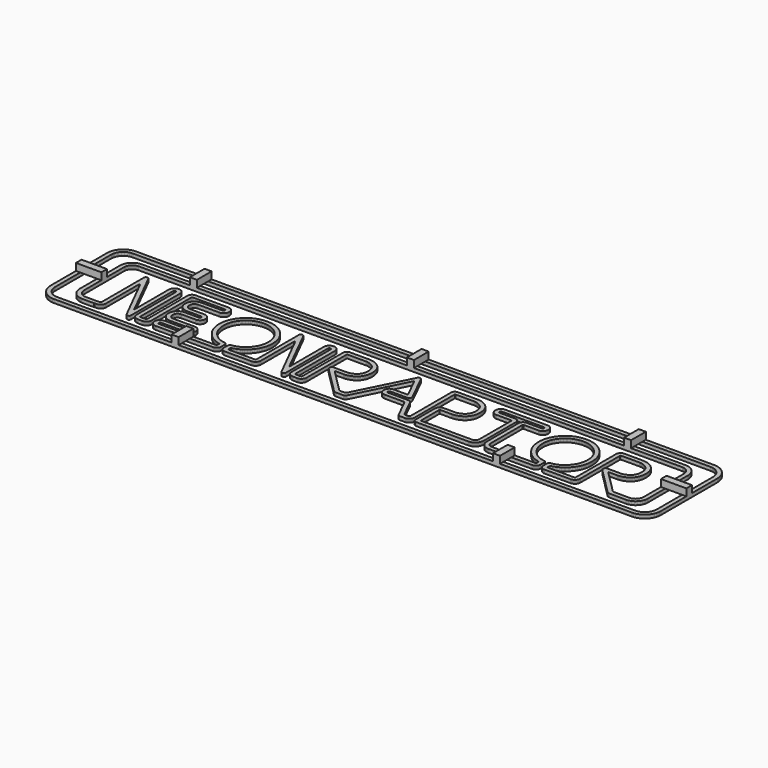
from build123d import *

# Parameters (mm, degrees)
F1_DEPTH = 2.5
F2_W     = 18.022328
F2_H     = 2.469339
F2_H_2   = 2.530661
F2_W_2   = 5
F2_H_3   = 13.05295
F2_H_4   = 13.02694
F2_W_3   = 18.022501
F2_H_5   = 5
F3_DEPTH = 5


with BuildPart() as f1:
    # F0 (on Top) → F1 (new body)
    with BuildSketch(Plane.XY):
        Polygon((206.175417, 36.451578), (205.000149, 36.511122), (-205.000148, 36.511122), (-206.175417, 36.45158), (-207.317119, 36.276841), (-208.419424, 35.992736), (-209.476501, 35.605094), (-210.482519, 35.119749), (-211.431648, 34.542529), (-212.318056, 33.879266), (-213.135913, 33.13579), (-213.879389, 32.317933), (-214.542652, 31.431524), (-215.119872, 30.482395), (-215.605218, 29.476377), (-215.992859, 28.4193), (-216.276964, 27.316995), (-216.451704, 26.175293), (-216.511246, 25.000025), (-216.511246, -25.000369), (-216.451704, -26.175633), (-216.276965, -27.317324), (-215.99286, -28.419612), (-215.605221, -29.476667), (-215.119877, -30.482659), (-214.542661, -31.431759), (-213.879403, -32.318136), (-213.135935, -33.135962), (-212.318087, -33.879405), (-211.43169, -34.542637), (-210.482575, -35.119828), (-209.476573, -35.605148), (-208.419516, -35.992767), (-207.317234, -36.276855), (-206.175559, -36.451583), (-205.00032, -36.511122), (205.000149, -36.511122), (206.175417, -36.451579), (207.317119, -36.27684), (208.419424, -35.992735), (209.476501, -35.605094), (210.482519, -35.119748), (211.431648, -34.542528), (212.318057, -33.879265), (213.135914, -33.135789), (213.87939, -32.317932), (214.542653, -31.431523), (215.119873, -30.482395), (215.605219, -29.476377), (215.99286, -28.4193), (216.276965, -27.316995), (216.451704, -26.175293), (216.511246, -25.000024), (216.511246, 24.999853), (216.451704, 26.175123), (216.276965, 27.316831), (215.99286, 28.419144), (215.605219, 29.476232), (215.119873, 30.482263), (214.542653, 31.431406), (213.87939, 32.31783), (213.135914, 33.135704), (212.318057, 33.879196), (211.431648, 34.542474), (210.482519, 35.119709), (209.476501, 35.605068), (208.419424, 35.99272), (207.317119, 36.276834), align=None)
        Polygon((213.489209, 24.999853), (213.489209, -25.000024), (213.445298, -25.866741), (213.316432, -26.708705), (213.106912, -27.521616), (212.821038, -28.301174), (212.463109, -29.043079), (212.037426, -29.74303), (211.548289, -30.396729), (210.999998, -30.999873), (210.396853, -31.548164), (209.743155, -32.037301), (209.043203, -32.462984), (208.301298, -32.820913), (207.52174, -33.106788), (206.708829, -33.316308), (205.866865, -33.445173), (205.000149, -33.489084), (-205.000148, -33.489084), (-205.866833, -33.445173), (-206.708764, -33.316308), (-207.521644, -33.106788), (-208.301171, -32.820913), (-209.043047, -32.462984), (-209.74297, -32.037301), (-210.396641, -31.548164), (-210.99976, -30.999873), (-211.548028, -30.396729), (-212.037144, -29.74303), (-212.462809, -29.043079), (-212.820722, -28.301174), (-213.106584, -27.521616), (-213.316095, -26.708705), (-213.444955, -25.866741), (-213.488863, -25.000024), (-213.488863, 25.000025), (-213.444955, 25.866709), (-213.316095, 26.708641), (-213.106584, 27.521521), (-212.820722, 28.301048), (-212.462809, 29.042923), (-212.037144, 29.742846), (-211.548028, 30.396518), (-210.99976, 30.999637), (-210.396641, 31.547905), (-209.74297, 32.037021), (-209.043047, 32.462686), (-208.301171, 32.820599), (-207.521644, 33.106461), (-206.708764, 33.315972), (-205.866833, 33.444831), (-205.000148, 33.48874), (205.000149, 33.48874), (205.866865, 33.444831), (206.708829, 33.315971), (207.52174, 33.10646), (208.301298, 32.820596), (209.043203, 32.46268), (209.743155, 32.037012), (210.396853, 31.54789), (210.999998, 30.999615), (211.548289, 30.396487), (212.037426, 29.742804), (212.463109, 29.042867), (212.821038, 28.300975), (213.106912, 27.521428), (213.316432, 26.708526), (213.445298, 25.866567), align=None, mode=Mode.SUBTRACT)
    extrude(amount=-F1_DEPTH)



with BuildPart() as f1b:
    # F0 (on Top) → F1, piece 2 (new body)
    with BuildSketch(Plane.XY):
        Polygon((193.738901, 26.435439), (192.855154, 26.48021), (-192.855498, 26.48021), (-193.739213, 26.435439), (-194.597688, 26.304049), (-195.426538, 26.090424), (-196.22138, 25.798948), (-196.977829, 25.434004), (-197.6915, 24.999977), (-198.35801, 24.50125), (-198.972975, 23.942208), (-199.53201, 23.327234), (-200.030731, 22.660713), (-200.464755, 21.947027), (-200.829696, 21.190562), (-201.121171, 20.395701), (-201.334795, 19.566827), (-201.466185, 18.708326), (-201.510955, 17.82458), (-201.510955, -17.885902), (-201.466185, -18.76965), (-201.334795, -19.628157), (-201.121171, -20.457039), (-200.829696, -21.251911), (-200.464755, -22.008389), (-200.030731, -22.722089), (-199.53201, -23.388626), (-198.972975, -24.003616), (-198.35801, -24.562675), (-197.6915, -25.061417), (-196.977829, -25.495458), (-196.22138, -25.860415), (-195.426538, -26.151902), (-194.597688, -26.365536), (-193.739213, -26.496932), (-192.855498, -26.541704), (-184.492184, -26.541704), (-184.392276, -26.441797), (-184.392276, -26.435595), (-183.063675, -26.435595), (-182.850104, -26.431205), (-182.641303, -26.418045), (-182.43731, -26.396129), (-182.238163, -26.365472), (-182.0439, -26.326088), (-181.854558, -26.277992), (-181.670178, -26.2212), (-181.490795, -26.155724), (-181.316449, -26.081581), (-181.147177, -25.998785), (-180.983018, -25.90735), (-180.82401, -25.807291), (-180.670191, -25.698622), (-180.521598, -25.581359), (-180.378271, -25.455516), (-180.240247, -25.321107), (-180.109215, -25.179928), (-179.986528, -25.033659), (-179.872199, -24.882341), (-179.766245, -24.72601), (-179.66868, -24.564705), (-179.579519, -24.398465), (-179.498778, -24.227327), (-179.426472, -24.051331), (-179.362616, -23.870514), (-179.307225, -23.684915), (-179.260314, -23.494573), (-179.221898, -23.299525), (-179.191993, -23.09981), (-179.170613, -22.895466), (-179.157775, -22.686532), (-179.153492, -22.473047), (-179.153492, 6.310037), (-179.150846, 6.362352), (-179.14315, 6.41153), (-179.130759, 6.457537), (-179.114034, 6.500341), (-179.093333, 6.539909), (-179.069013, 6.576209), (-179.041433, 6.609208), (-179.010951, 6.638872), (-178.977925, 6.665169), (-178.942715, 6.688066), (-178.905678, 6.70753), (-178.867172, 6.723529), (-178.827556, 6.73603), (-178.787188, 6.745), (-178.746426, 6.750406), (-178.705629, 6.752215), (-178.674337, 6.751181), (-178.643736, 6.748101), (-178.613879, 6.743008), (-178.584819, 6.735934), (-178.556609, 6.726914), (-178.529301, 6.71598), (-178.50295, 6.703165), (-178.477607, 6.688503), (-178.453326, 6.672025), (-178.430159, 6.653766), (-178.408161, 6.633758), (-178.387383, 6.612035), (-178.367879, 6.588629), (-178.349702, 6.563574), (-178.332904, 6.536902), (-178.317539, 6.508647), (-162.067713, -25.757945), (-162.025939, -25.832576), (-161.977046, -25.905069), (-161.921637, -25.975056), (-161.86031, -26.042165), (-161.793667, -26.106029), (-161.722309, -26.166278), (-161.646837, -26.222541), (-161.567851, -26.274451), (-161.485952, -26.321637), (-161.401741, -26.36373), (-161.315819, -26.400361), (-161.228786, -26.43116), (-161.141244, -26.455758), (-161.053793, -26.473785), (-160.967033, -26.484872), (-160.881566, -26.48865), (-160.612677, -26.48865), (-160.485065, -26.482187), (-160.361098, -26.463219), (-160.241408, -26.432378), (-160.12663, -26.390298), (-160.017396, -26.337609), (-159.914339, -26.274946), (-159.818093, -26.202939), (-159.72929, -26.122221), (-159.648563, -26.033425), (-159.576546, -25.937182), (-159.513871, -25.834126), (-159.461172, -25.724888), (-159.419082, -25.610101), (-159.388234, -25.490398), (-159.369261, -25.36641), (-159.362796, -25.238769), (-159.362796, 11.975841), (-159.359311, 12.100918), (-159.348815, 12.217424), (-159.331244, 12.325429), (-159.306533, 12.425001), (-159.274621, 12.51621), (-159.235442, 12.599126), (-159.188934, 12.673816), (-159.135032, 12.740351), (-159.073674, 12.798799), (-159.004795, 12.84923), (-158.928333, 12.891713), (-158.844223, 12.926316), (-158.752402, 12.95311), (-158.652806, 12.972162), (-158.545372, 12.983543), (-158.430036, 12.987321), (-158.308364, 12.983549), (-158.195029, 12.972187), (-158.089965, 12.953165), (-157.993104, 12.926416), (-157.904379, 12.891869), (-157.823723, 12.849457), (-157.751069, 12.79911), (-157.686348, 12.74076), (-157.629494, 12.674337), (-157.580439, 12.599773), (-157.539115, 12.516999), (-157.505456, 12.425946), (-157.479394, 12.326544), (-157.460862, 12.218726), (-157.449792, 12.102422), (-157.446117, 11.977564), (-157.446117, -22.425849), (-157.430749, -22.85257), (-157.384663, -23.255621), (-157.307892, -23.634948), (-157.200466, -23.990498), (-157.062415, -24.322219), (-156.893771, -24.630056), (-156.694564, -24.913959), (-156.464825, -25.173872), (-156.204585, -25.409744), (-155.913874, -25.621521), (-155.592724, -25.809151), (-155.241165, -25.97258), (-154.859227, -26.111755), (-154.446943, -26.226624), (-154.004342, -26.317133), (-153.531455, -26.38323), (-150.626206, -26.48865), (-150.412654, -26.48426), (-150.20365, -26.4711), (-149.999235, -26.449185), (-149.799448, -26.418531), (-149.604327, -26.379153), (-149.413913, -26.331065), (-149.228245, -26.274283), (-149.047362, -26.208822), (-148.871303, -26.134697), (-148.700108, -26.051923), (-148.533817, -25.960516), (-148.372468, -25.86049), (-148.216101, -25.751861), (-148.064755, -25.634644), (-147.91847, -25.508854), (-147.777284, -25.374506), (-147.642967, -25.233383), (-147.517203, -25.087156), (-147.400009, -24.935863), (-147.291399, -24.779543), (-147.19139, -24.618236), (-147.099997, -24.451979), (-147.017235, -24.280812), (-146.943119, -24.104773), (-146.877665, -23.923902), (-146.820889, -23.738237), (-146.772805, -23.547817), (-146.733429, -23.352682), (-146.702776, -23.152869), (-146.680862, -22.948418), (-146.667703, -22.739367), (-146.663313, -22.525756), (-146.663313, 12.154297), (-146.658731, 12.244721), (-146.645284, 12.332564), (-146.62342, 12.417377), (-146.59359, 12.498713), (-146.556241, 12.576121), (-146.511823, 12.649153), (-146.460784, 12.71736), (-146.403574, 12.780293), (-146.340641, 12.837503), (-146.272434, 12.888542), (-146.199402, 12.93296), (-146.121994, 12.970308), (-146.040659, 13.000139), (-145.955845, 13.022002), (-145.868002, 13.035449), (-145.777579, 13.040031), (-123.479887, 13.040031), (-123.354841, 13.036451), (-123.238361, 13.025668), (-123.13038, 13.007616), (-123.030827, 12.982229), (-122.939634, 12.949442), (-122.856733, 12.909189), (-122.782054, 12.861405), (-122.715528, 12.806023), (-122.657087, 12.742979), (-122.606661, 12.672207), (-122.564183, 12.593641), (-122.529582, 12.507215), (-122.50279, 12.412864), (-122.483738, 12.310523), (-122.472358, 12.200125), (-122.468579, 12.081606), (-122.472358, 11.963115), (-122.483738, 11.852738), (-122.50279, 11.750411), (-122.529582, 11.656069), (-122.564183, 11.569647), (-122.606661, 11.49108), (-122.657087, 11.420304), (-122.715528, 11.357253), (-122.782054, 11.301862), (-122.856733, 11.254068), (-122.939634, 11.213804), (-123.030827, 11.181007), (-123.13038, 11.15561), (-123.238361, 11.13755), (-123.354841, 11.126762), (-123.479887, 11.12318), (-138.296554, 11.12318), (-138.640569, 11.115978), (-138.977524, 11.094387), (-139.307355, 11.058432), (-139.63, 11.008138), (-139.945393, 10.943529), (-140.253472, 10.864629), (-140.554173, 10.771464), (-140.847432, 10.664057), (-141.133186, 10.542432), (-141.411371, 10.406615), (-141.681924, 10.25663), (-141.944781, 10.092502), (-142.199878, 9.914254), (-142.447152, 9.721911), (-142.68654, 9.515499), (-142.917977, 9.29504), (-143.13847, 9.063512), (-143.34492, 8.824045), (-143.537303, 8.576703), (-143.715592, 8.321548), (-143.879764, 8.058643), (-144.029792, 7.788053), (-144.165651, 7.509838), (-144.287317, 7.224064), (-144.394763, 6.930793), (-144.487965, 6.630087), (-144.566898, 6.322011), (-144.631535, 6.006627), (-144.681853, 5.683998), (-144.717826, 5.354187), (-144.739428, 5.017257), (-144.746634, 4.673272), (-144.739428, 4.329166), (-144.717826, 3.992133), (-144.681854, 3.662236), (-144.631538, 3.339539), (-144.566903, 3.024106), (-144.487974, 2.716), (-144.394777, 2.415287), (-144.287338, 2.122028), (-144.165682, 1.83629), (-144.029834, 1.558134), (-143.87982, 1.287625), (-143.715665, 1.024827), (-143.537395, 0.769804), (-143.345035, 0.52262), (-143.138612, 0.283337), (-142.918149, 0.052021), (-142.686805, -0.1685), (-142.447501, -0.374971), (-142.2003, -0.567368), (-141.945265, -0.745666), (-141.682459, -0.909841), (-141.411943, -1.059869), (-141.133781, -1.195724), (-140.848035, -1.317383), (-140.554767, -1.42482), (-140.254041, -1.518012), (-139.945919, -1.596934), (-139.630463, -1.661561), (-139.307735, -1.711869), (-138.9778, -1.747834), (-138.640719, -1.769431), (-138.296554, -1.776635), (-128.401206, -1.776635), (-128.282687, -1.78012), (-128.172289, -1.790616), (-128.069948, -1.808187), (-127.975597, -1.832895), (-127.889171, -1.864806), (-127.810605, -1.90398), (-127.739833, -1.950483), (-127.676789, -2.004378), (-127.621407, -2.065727), (-127.573623, -2.134594), (-127.53337, -2.211042), (-127.500583, -2.295136), (-127.475196, -2.386937), (-127.457144, -2.48651), (-127.44636, -2.593917), (-127.442781, -2.709223), (-127.44636, -2.830928), (-127.457144, -2.944295), (-127.475196, -3.04939), (-127.500583, -3.146282), (-127.53337, -3.235036), (-127.573623, -3.31572), (-127.621407, -3.388402), (-127.676789, -3.453148), (-127.739833, -3.510026), (-127.810605, -3.559102), (-127.889171, -3.600443), (-127.975597, -3.634118), (-128.069948, -3.660192), (-128.172289, -3.678734), (-128.282687, -3.68981), (-128.401206, -3.693487), (-138.296554, -3.693487), (-138.640599, -3.700644), (-138.97758, -3.722102), (-139.307433, -3.757834), (-139.630094, -3.807815), (-139.945499, -3.872022), (-140.253584, -3.950429), (-140.554285, -4.043012), (-140.847539, -4.149746), (-141.133282, -4.270607), (-141.41145, -4.405568), (-141.681979, -4.554607), (-141.944805, -4.717697), (-142.199865, -4.894815), (-142.447094, -5.085936), (-142.686428, -5.291034), (-142.917805, -5.510085), (-143.138328, -5.740294), (-143.344805, -5.978708), (-143.53721, -6.225266), (-143.71552, -6.479907), (-143.879708, -6.742567), (-144.02975, -7.013185), (-144.16562, -7.291699), (-144.287295, -7.578047), (-144.394749, -7.872166), (-144.487956, -8.173995), (-144.566892, -8.483472), (-144.631533, -8.800534), (-144.681852, -9.125119), (-144.717825, -9.457166), (-144.739428, -9.796611), (-144.746634, -10.143394), (-144.73943, -10.490342), (-144.717833, -10.830154), (-144.68187, -11.162765), (-144.631565, -11.488112), (-144.566943, -11.806131), (-144.488029, -12.11676), (-144.394847, -12.419933), (-144.287424, -12.715589), (-144.165784, -13.003662), (-144.029951, -13.28409), (-143.879952, -13.556809), (-143.71581, -13.821755), (-143.537551, -14.078865), (-143.3452, -14.328075), (-143.138782, -14.569322), (-142.918322, -14.802541), (-142.687006, -15.024847), (-142.447722, -15.232989), (-142.200535, -15.426944), (-141.945508, -15.606686), (-141.682702, -15.772191), (-141.412182, -15.923434), (-141.13401, -16.06039), (-140.84825, -16.183034), (-140.554964, -16.291343), (-140.254217, -16.38529), (-139.94607, -16.464852), (-139.630586, -16.530004), (-139.30783, -16.58072), (-138.977864, -16.616977), (-138.640751, -16.638749), (-138.296554, -16.646012), (-123.479887, -16.646012), (-123.354841, -16.649689), (-123.238361, -16.660765), (-123.13038, -16.679306), (-123.030827, -16.705381), (-122.939634, -16.739055), (-122.856733, -16.780397), (-122.782054, -16.829473), (-122.715528, -16.88635), (-122.657087, -16.951096), (-122.606661, -17.023778), (-122.564183, -17.104463), (-122.529582, -17.193217), (-122.50279, -17.290108), (-122.483738, -17.395204), (-122.472358, -17.508571), (-122.468579, -17.630276), (-122.472358, -17.74561), (-122.483738, -17.853038), (-122.50279, -17.952625), (-122.529582, -18.044435), (-122.564183, -18.128532), (-122.606661, -18.20498), (-122.657087, -18.273843), (-122.715528, -18.335185), (-122.782054, -18.389071), (-122.856733, -18.435564), (-122.939634, -18.474728), (-123.030827, -18.506627), (-123.13038, -18.531327), (-123.238361, -18.54889), (-123.354841, -18.55938), (-123.479887, -18.562863), (-140.730686, -18.562863), (-140.944125, -18.567249), (-141.153242, -18.580397), (-141.357997, -18.602291), (-141.558351, -18.632917), (-141.754266, -18.672259), (-141.945701, -18.720303), (-142.132618, -18.777032), (-142.314978, -18.842433), (-142.492741, -18.916489), (-142.665869, -18.999186), (-142.834323, -19.090508), (-142.998062, -19.190441), (-143.157049, -19.298969), (-143.311244, -19.416077), (-143.460608, -19.541751), (-143.605102, -19.675973), (-143.742738, -19.817221), (-143.87161, -19.963566), (-143.991701, -20.114968), (-144.102996, -20.271388), (-144.205479, -20.432789), (-144.299133, -20.599131), (-144.383944, -20.770374), (-144.459894, -20.946482), (-144.526969, -21.127413), (-144.585152, -21.313131), (-144.634428, -21.503595), (-144.674779, -21.698767), (-144.706192, -21.898608), (-144.728649, -22.103079), (-144.742135, -22.312141), (-144.746634, -22.525756), (-144.742135, -22.739553), (-144.728649, -22.948773), (-144.706192, -23.153378), (-144.674779, -23.353328), (-144.634428, -23.548584), (-144.585152, -23.739109), (-144.526969, -23.924863), (-144.459894, -24.105806), (-144.383944, -24.281902), (-144.299133, -24.453109), (-144.205479, -24.61939), (-144.102996, -24.780706), (-143.991701, -24.937018), (-143.87161, -25.088286), (-143.742738, -25.234473), (-143.605102, -25.375539), (-143.460818, -25.509762), (-143.311633, -25.635436), (-143.157585, -25.752544), (-142.998716, -25.861072), (-142.835065, -25.961005), (-142.666672, -26.052327), (-142.493576, -26.135024), (-142.315818, -26.20908), (-142.133437, -26.274481), (-141.946473, -26.33121), (-141.754967, -26.379254), (-141.558957, -26.418596), (-141.358484, -26.449222), (-141.153588, -26.471116), (-140.944309, -26.484264), (-140.730686, -26.48865), (-100.001561, -26.48865), (-99.681719, -26.472446), (-99.371012, -26.424894), (-99.071028, -26.347579), (-98.783354, -26.242089), (-98.509576, -26.110009), (-98.251281, -25.952927), (-98.010055, -25.772429), (-97.787485, -25.570101), (-97.585157, -25.347531), (-97.404659, -25.106305), (-97.247577, -24.84801), (-97.115497, -24.574232), (-97.010007, -24.286558), (-96.932692, -23.986574), (-96.88514, -23.675867), (-96.868936, -23.356024), (-96.868936, -19.837204), (-96.875413, -19.698053), (-96.894474, -19.56214), (-96.925567, -19.430095), (-96.968139, -19.302547), (-97.021638, -19.180126), (-97.085511, -19.063462), (-97.159206, -18.953186), (-97.242169, -18.849926), (-97.333849, -18.754312), (-97.433693, -18.666975), (-97.541148, -18.588544), (-97.655661, -18.519649), (-97.776681, -18.460919), (-97.903654, -18.412985), (-98.036027, -18.376477), (-98.173249, -18.352023), (-98.892341, -18.245388), (-99.597226, -18.108596), (-100.287771, -17.941719), (-100.963844, -17.744831), (-101.625311, -17.518004), (-102.272039, -17.261313), (-102.903896, -16.974831), (-103.520748, -16.65863), (-104.122463, -16.312783), (-104.708907, -15.937365), (-105.279947, -15.532447), (-105.835451, -15.098104), (-106.375286, -14.634408), (-106.899318, -14.141432), (-107.407415, -13.619251), (-107.899443, -13.067936), (-108.368725, -12.496431), (-108.808118, -11.913466), (-109.217569, -11.319186), (-109.597024, -10.713735), (-109.946431, -10.097256), (-110.265735, -9.469894), (-110.554883, -8.831791), (-110.813821, -8.183092), (-111.042497, -7.523941), (-111.240856, -6.854481), (-111.408845, -6.174856), (-111.54641, -5.485211), (-111.653499, -4.785688), (-111.730057, -4.076432), (-111.776031, -3.357587), (-111.791367, -2.629297), (-111.773132, -1.811912), (-111.718467, -1.008791), (-111.627436, -0.220088), (-111.500103, 0.554044), (-111.336531, 1.313452), (-111.136783, 2.057981), (-110.900923, 2.787478), (-110.629014, 3.501789), (-110.321118, 4.200761), (-109.977301, 4.88424), (-109.597624, 5.552072), (-109.182152, 6.204103), (-108.730947, 6.840181), (-108.244073, 7.46015), (-107.721593, 8.063859), (-107.16357, 8.651152), (-106.579594, 9.212273), (-105.978988, 9.737653), (-105.361907, 10.227229), (-104.728504, 10.680938), (-104.078933, 11.098715), (-103.413348, 11.480497), (-102.731902, 11.826221), (-102.034749, 12.135823), (-101.322043, 12.409239), (-100.593937, 12.646406), (-99.850584, 12.847261), (-99.09214, 13.011738), (-98.318756, 13.139776), (-97.530588, 13.231311), (-96.727788, 13.286278), (-95.910511, 13.304615), (-95.087056, 13.286379), (-94.278453, 13.231715), (-93.484855, 13.140686), (-92.706418, 13.013356), (-91.943298, 12.849789), (-91.195649, 12.650049), (-90.463626, 12.414199), (-89.747385, 12.142304), (-89.047082, 11.834427), (-88.36287, 11.490632), (-87.694905, 11.110983), (-87.043344, 10.695544), (-86.408339, 10.244379), (-85.790048, 9.757551), (-85.188624, 9.235124), (-84.604224, 8.677162), (-84.046234, 8.092732), (-83.523786, 7.491282), (-83.036944, 6.872967), (-82.585769, 6.237943), (-82.170327, 5.586365), (-81.790678, 4.918386), (-81.446888, 4.234163), (-81.139018, 3.53385), (-80.867131, 2.817602), (-80.631292, 2.085574), (-80.431563, 1.337921), (-80.268006, 0.574798), (-80.140686, -0.20364), (-80.049664, -0.997238), (-79.995005, -1.805842), (-79.976772, -2.629297), (-79.992161, -3.357345), (-80.038293, -4.07598), (-80.115115, -4.785058), (-80.222574, -5.484436), (-80.360617, -6.173968), (-80.529191, -6.853512), (-80.728243, -7.522923), (-80.95772, -8.182058), (-81.217569, -8.830773), (-81.507736, -9.468925), (-81.82817, -10.096368), (-82.178818, -10.71296), (-82.559625, -11.318557), (-82.970539, -11.913014), (-83.411507, -12.496188), (-83.882476, -13.067936), (-84.376399, -13.619251), (-84.886436, -14.141433), (-85.41246, -14.63441), (-85.954343, -15.098109), (-86.511959, -15.532458), (-87.085179, -15.937383), (-87.673876, -16.312812), (-88.277923, -16.658673), (-88.897192, -16.974892), (-89.531557, -17.261398), (-90.180888, -17.518116), (-90.84506, -17.744976), (-91.523945, -17.941904), (-92.217414, -18.108826), (-92.925342, -18.245672), (-93.6476, -18.352368), (-93.784823, -18.376765), (-93.917203, -18.413232), (-94.044184, -18.461138), (-94.165214, -18.519853), (-94.279741, -18.588746), (-94.38721, -18.667186), (-94.48707, -18.754543), (-94.578766, -18.850184), (-94.661746, -18.95348), (-94.735456, -19.0638), (-94.799343, -19.180513), (-94.852856, -19.302988), (-94.895439, -19.430594), (-94.92654, -19.562701), (-94.945607, -19.698678), (-94.952085, -19.837893), (-94.952085, -23.356024), (-94.935882, -23.675867), (-94.888329, -23.986574), (-94.811012, -24.286558), (-94.705518, -24.574232), (-94.573434, -24.84801), (-94.416344, -25.106305), (-94.235835, -25.347531), (-94.033493, -25.570101), (-93.810905, -25.772429), (-93.569656, -25.952927), (-93.311333, -26.110009), (-93.037522, -26.242089), (-92.749808, -26.347579), (-92.449778, -26.424894), (-92.139019, -26.472446), (-91.819115, -26.48865), (-73.103462, -26.435595), (-72.889919, -26.431205), (-72.68114, -26.418045), (-72.477162, -26.396129), (-72.278025, -26.365472), (-72.083768, -26.326088), (-71.89443, -26.277992), (-71.71005, -26.2212), (-71.530668, -26.155724), (-71.356322, -26.081581), (-71.187052, -25.998785), (-71.022896, -25.90735), (-70.863894, -25.807291), (-70.710085, -25.698622), (-70.561508, -25.581359), (-70.418202, -25.455516), (-70.280206, -25.321107), (-70.149146, -25.179984), (-70.026437, -25.033758), (-69.912094, -24.882469), (-69.806131, -24.726155), (-69.708563, -24.564858), (-69.619403, -24.398616), (-69.538666, -24.22747), (-69.466367, -24.05146), (-69.402519, -23.870625), (-69.347139, -23.685006), (-69.300238, -23.494642), (-69.261833, -23.299573), (-69.231937, -23.09984), (-69.210565, -22.89548), (-69.197732, -22.686536), (-69.193451, -22.473047), (-69.193451, 6.619751), (-69.191246, 6.663351), (-69.184829, 6.704342), (-69.1745, 6.742697), (-69.160555, 6.778387), (-69.143294, 6.811385), (-69.123015, 6.841661), (-69.100016, 6.869188), (-69.074595, 6.893938), (-69.04705, 6.915882), (-69.01768, 6.934991), (-68.986783, 6.951238), (-68.954657, 6.964595), (-68.921601, 6.975032), (-68.887912, 6.982523), (-68.853889, 6.987038), (-68.81983, 6.988549), (-68.793809, 6.987685), (-68.768358, 6.985114), (-68.74352, 6.980862), (-68.719341, 6.974957), (-68.695864, 6.967427), (-68.673134, 6.9583), (-68.651195, 6.947603), (-68.630091, 6.935365), (-68.609868, 6.921613), (-68.59057, 6.906375), (-68.57224, 6.889678), (-68.554924, 6.87155), (-68.538665, 6.85202), (-68.523509, 6.831114), (-68.509499, 6.808861), (-68.49668, 6.785288), (-52.193971, -25.586379), (-52.138186, -25.688258), (-52.07614, -25.78499), (-52.008153, -25.876379), (-51.934545, -25.962228), (-51.855636, -26.042341), (-51.771747, -26.116519), (-51.683196, -26.184567), (-51.590305, -26.246287), (-51.493392, -26.301484), (-51.392778, -26.349959), (-51.288783, -26.391517), (-51.181727, -26.42596), (-51.07193, -26.453091), (-50.959711, -26.472715), (-50.845391, -26.484633), (-50.729289, -26.48865), (-50.593831, -26.481789), (-50.462243, -26.461656), (-50.335196, -26.42892), (-50.213362, -26.384253), (-50.097413, -26.328326), (-49.988022, -26.26181), (-49.88586, -26.185378), (-49.791599, -26.099699), (-49.705911, -26.005444), (-49.629468, -25.903286), (-49.562941, -25.793896), (-49.507004, -25.677943), (-49.462328, -25.556101), (-49.429584, -25.429039), (-49.409445, -25.29743), (-49.402583, -25.161944), (-49.402583, 11.975841), (-49.399098, 12.100918), (-49.388602, 12.217424), (-49.37103, 12.325429), (-49.34632, 12.425001), (-49.314407, 12.51621), (-49.275229, 12.599126), (-49.22872, 12.673816), (-49.174819, 12.740351), (-49.113461, 12.798799), (-49.044582, 12.84923), (-48.96812, 12.891713), (-48.88401, 12.926316), (-48.792189, 12.95311), (-48.692593, 12.972162), (-48.585159, 12.983543), (-48.469823, 12.987321), (-48.34815, 12.983549), (-48.234816, 12.972187), (-48.129752, 12.953165), (-48.032891, 12.926416), (-47.944166, 12.891869), (-47.86351, 12.849457), (-47.790856, 12.79911), (-47.726135, 12.74076), (-47.66928, 12.674337), (-47.620225, 12.599773), (-47.578902, 12.516999), (-47.545243, 12.425946), (-47.519181, 12.326544), (-47.500649, 12.218726), (-47.489579, 12.102422), (-47.485904, 11.977564), (-47.485904, -22.425849), (-47.470535, -22.852627), (-47.42445, -23.25572), (-47.347679, -23.635076), (-47.240252, -23.990643), (-47.102202, -24.322371), (-46.933558, -24.630208), (-46.734351, -24.914102), (-46.504612, -25.174001), (-46.244371, -25.409855), (-45.953661, -25.621612), (-45.63251, -25.80922), (-45.280951, -25.972628), (-44.899014, -26.111785), (-44.48673, -26.226638), (-44.044129, -26.317137), (-43.571242, -26.38323), (-40.665993, -26.48865), (-40.452441, -26.48426), (-40.243437, -26.4711), (-40.039022, -26.449185), (-39.839235, -26.418531), (-39.644114, -26.379153), (-39.4537, -26.331065), (-39.268032, -26.274283), (-39.087149, -26.208822), (-38.91109, -26.134697), (-38.739895, -26.051923), (-38.573604, -25.960516), (-38.412255, -25.86049), (-38.255887, -25.751861), (-38.104542, -25.634644), (-37.958256, -25.508854), (-37.817071, -25.374506), (-37.682753, -25.233383), (-37.55699, -25.087156), (-37.439796, -24.935863), (-37.331186, -24.779543), (-37.231177, -24.618236), (-37.139784, -24.451979), (-37.057022, -24.280812), (-36.982906, -24.104773), (-36.917452, -23.923902), (-36.860675, -23.738237), (-36.812591, -23.547817), (-36.773215, -23.352682), (-36.742563, -23.152869), (-36.720649, -22.948418), (-36.70749, -22.739367), (-36.7031, -22.525756), (-36.7031, 12.265574), (-36.699093, 12.344642), (-36.687337, 12.421453), (-36.668221, 12.495613), (-36.64214, 12.566732), (-36.609485, 12.634415), (-36.570649, 12.698272), (-36.526025, 12.757909), (-36.476003, 12.812935), (-36.420978, 12.862956), (-36.36134, 12.907581), (-36.297484, 12.946417), (-36.2298, 12.979072), (-36.158682, 13.005153), (-36.084521, 13.024268), (-36.00771, 13.036025), (-35.928642, 13.040031), (-23.088701, 13.035696), (-22.815225, 13.0227), (-22.541772, 13.00106), (-22.268402, 12.97079), (-21.995176, 12.931907), (-21.722154, 12.884427), (-21.449394, 12.828364), (-21.176959, 12.763735), (-20.904906, 12.690555), (-20.633298, 12.608839), (-20.362193, 12.518604), (-20.091651, 12.419866), (-19.821734, 12.312639), (-19.5525, 12.196939), (-19.28401, 12.072782), (-19.016324, 11.940185), (-18.531485, 11.667832), (-18.077526, 11.37077), (-17.654501, 11.0491), (-17.262466, 10.702919), (-16.901477, 10.332328), (-16.571588, 9.937427), (-16.272854, 9.518315), (-16.005332, 9.075092), (-15.769076, 8.607858), (-15.564141, 8.116712), (-15.390584, 7.601754), (-15.248458, 7.063084), (-15.13782, 6.500801), (-15.058724, 5.915005), (-15.011226, 5.305795), (-14.995381, 4.673272), (-15.011225, 4.0406), (-15.058722, 3.431266), (-15.137815, 2.845369), (-15.248447, 2.283011), (-15.390563, 1.744291), (-15.564105, 1.229309), (-15.769018, 0.738164), (-16.005246, 0.270957), (-16.272732, -0.172212), (-16.571419, -0.591244), (-16.901253, -0.986038), (-17.262175, -1.356495), (-17.654131, -1.702515), (-18.077064, -2.023997), (-18.530917, -2.320843), (-19.015635, -2.592951), (-19.295556, -2.731996), (-19.574654, -2.862188), (-19.852869, -2.98351), (-20.130142, -3.095945), (-20.406413, -3.199479), (-20.681621, -3.294095), (-20.955708, -3.379776), (-21.228613, -3.456507), (-21.500277, -3.524271), (-21.77064, -3.583052), (-22.039641, -3.632835), (-22.307222, -3.673602), (-22.573322, -3.705338), (-22.837881, -3.728026), (-23.10084, -3.741651), (-33.039585, -3.746196), (-33.158492, -3.752223), (-33.274006, -3.769907), (-33.385538, -3.79866), (-33.492497, -3.83789), (-33.594292, -3.887007), (-33.690333, -3.945421), (-33.780029, -4.012542), (-33.862791, -4.087778), (-33.938027, -4.170539), (-34.005147, -4.260236), (-34.063561, -4.356277), (-34.112678, -4.458072), (-34.151909, -4.56503), (-34.180661, -4.676562), (-34.198346, -4.792076), (-34.204372, -4.910983), (-34.204372, -5.738495), (-34.202298, -5.82046), (-34.19612, -5.902047), (-34.185907, -5.983095), (-34.171724, -6.063443), (-34.15364, -6.142931), (-34.13172, -6.221399), (-34.106033, -6.298686), (-34.076645, -6.374632), (-34.043624, -6.449076), (-34.007036, -6.521857), (-33.966949, -6.592816), (-33.92343, -6.661792), (-33.876546, -6.728623), (-33.826363, -6.793151), (-33.772951, -6.855213), (-33.716374, -6.914651), (-14.917177, -25.664238), (-14.815132, -25.761098), (-14.709176, -25.852283), (-14.599501, -25.937715), (-14.486298, -26.017312), (-14.369758, -26.090998), (-14.250073, -26.158691), (-14.127433, -26.220314), (-14.00203, -26.275786), (-13.874056, -26.325029), (-13.743701, -26.367963), (-13.611158, -26.404509), (-13.476616, -26.434589), (-13.340267, -26.458122), (-13.202303, -26.475029), (-13.062915, -26.485231), (-12.922294, -26.48865), (-7.661461, -26.48865), (-7.531059, -26.484129), (-7.402671, -26.470714), (-7.276659, -26.448627), (-7.153382, -26.41809), (-7.033201, -26.379325), (-6.916476, -26.332555), (-6.803566, -26.278), (-6.694832, -26.215884), (-6.590634, -26.146429), (-6.491332, -26.069855), (-6.397285, -25.986387), (-6.308855, -25.896244), (-6.226401, -25.79965), (-6.150283, -25.696827), (-6.080861, -25.587996), (-6.018495, -25.47338), (12.185389, 10.934561), (12.193933, 10.950393), (12.20339, 10.965381), (12.213718, 10.9795), (12.224879, 10.992727), (12.23683, 11.005036), (12.249533, 11.016403), (12.262946, 11.026803), (12.277029, 11.036213), (12.291742, 11.044607), (12.307044, 11.051962), (12.322896, 11.058252), (12.339256, 11.063453), (12.356084, 11.067542), (12.373341, 11.070492), (12.390985, 11.07228), (12.408976, 11.072882), (12.426967, 11.07228), (12.444611, 11.070492), (12.461868, 11.067542), (12.478696, 11.063453), (12.495056, 11.058252), (12.510908, 11.051962), (12.52621, 11.044607), (12.540923, 11.036213), (12.555006, 11.026803), (12.568419, 11.016403), (12.581122, 11.005036), (12.593073, 10.992727), (12.604233, 10.9795), (12.614562, 10.965381), (12.624018, 10.950393), (12.632563, 10.934561), (19.736005, -3.272151), (19.742982, -3.287187), (19.748927, -3.302485), (19.753842, -3.318002), (19.757731, -3.333695), (19.760593, -3.349518), (19.762433, -3.365429), (19.76325, -3.381384), (19.763049, -3.397337), (19.76183, -3.413247), (19.759596, -3.429068), (19.756348, -3.444757), (19.752089, -3.46027), (19.746821, -3.475562), (19.740545, -3.490591), (19.733265, -3.505312), (19.724981, -3.519681), (19.715806, -3.533469), (19.705878, -3.546524), (19.695233, -3.558826), (19.683909, -3.570351), (19.671942, -3.58108), (19.659372, -3.590989), (19.646234, -3.600057), (19.632566, -3.608263), (19.618406, -3.615585), (19.60379, -3.622001), (19.588757, -3.62749), (19.573343, -3.632029), (19.557586, -3.635598), (19.541523, -3.638173), (19.525191, -3.639735), (19.508629, -3.64026), (9.921961, -3.64026), (9.702129, -3.644547), (9.487464, -3.657398), (9.278004, -3.678798), (9.07379, -3.708731), (8.87486, -3.747183), (8.681255, -3.794138), (8.493013, -3.849582), (8.310174, -3.913499), (8.132777, -3.985874), (7.960861, -4.066691), (7.794466, -4.155937), (7.633632, -4.253594), (7.478397, -4.35965), (7.328802, -4.474087), (7.184884, -4.596892), (7.046685, -4.728049), (6.91553, -4.866248), (6.792731, -5.010166), (6.678302, -5.159761), (6.572257, -5.314996), (6.474613, -5.47583), (6.385382, -5.642225), (6.30458, -5.81414), (6.232221, -5.991537), (6.16832, -6.174377), (6.112892, -6.362619), (6.065951, -6.556224), (6.027512, -6.755154), (5.99759, -6.959368), (5.976199, -7.168828), (5.963353, -7.383493), (5.959068, -7.603325), (5.963454, -7.816916), (5.976602, -8.026164), (5.998496, -8.231031), (6.029122, -8.431478), (6.068464, -8.627465), (6.116508, -8.818955), (6.173237, -9.005908), (6.238638, -9.188285), (6.312694, -9.366047), (6.395391, -9.539156), (6.486713, -9.707573), (6.586646, -9.871259), (6.695174, -10.030174), (6.812282, -10.184281), (6.937955, -10.33354), (7.072178, -10.477913), (7.213245, -10.615515), (7.359431, -10.744349), (7.5107, -10.864401), (7.667012, -10.975654), (7.828328, -11.078094), (7.994609, -11.171705), (8.165816, -11.256474), (8.341911, -11.332383), (8.522855, -11.399418), (8.708609, -11.457565), (8.899134, -11.506807), (9.09439, -11.547131), (9.29434, -11.57852), (9.498945, -11.600959), (9.708165, -11.614434), (9.921961, -11.618929), (23.495293, -11.618929), (23.539823, -11.620474), (23.583673, -11.62506), (23.626718, -11.632609), (23.668834, -11.643044), (23.7099, -11.65629), (23.749789, -11.672268), (23.78838, -11.690904), (23.825549, -11.712119), (23.861171, -11.735837), (23.895123, -11.761981), (23.927281, -11.790475), (23.957523, -11.821242), (23.985723, -11.854205), (24.011759, -11.889288), (24.035507, -11.926414), (24.056844, -11.965505), (30.986653, -25.775515), (31.030621, -25.856024), (31.079542, -25.932468), (31.133164, -26.004693), (31.191233, -26.072541), (31.253494, -26.135858), (31.319694, -26.194488), (31.389579, -26.248273), (31.462895, -26.297059), (31.539388, -26.34069), (31.618805, -26.379009), (31.700891, -26.411861), (31.785393, -26.439089), (31.872057, -26.460538), (31.96063, -26.476052), (32.050856, -26.485474), (32.142483, -26.48865), (35.956204, -26.48865), (36.169754, -26.48426), (36.378752, -26.4711), (36.583158, -26.449185), (36.782935, -26.418531), (36.978042, -26.379153), (37.168442, -26.331065), (37.354094, -26.274283), (37.534962, -26.208822), (37.711004, -26.134697), (37.882183, -26.051923), (38.048461, -25.960516), (38.209797, -25.86049), (38.366153, -25.751861), (38.51749, -25.634644), (38.66377, -25.508854), (38.804953, -25.374506), (38.939301, -25.233383), (39.065091, -25.087156), (39.182309, -24.935863), (39.290938, -24.779543), (39.390963, -24.618236), (39.48237, -24.451979), (39.565144, -24.280812), (39.639269, -24.104773), (39.70473, -23.923902), (39.761512, -23.738237), (39.8096, -23.547817), (39.848978, -23.352682), (39.879633, -23.152869), (39.901547, -22.948418), (39.914707, -22.739367), (39.919097, -22.525756), (39.919097, 12.543249), (39.921667, 12.593962), (39.929209, 12.64323), (39.941472, 12.690798), (39.958204, 12.736416), (39.979153, 12.779832), (40.004066, 12.820793), (40.032693, 12.859049), (40.064781, 12.894347), (40.100079, 12.926435), (40.138335, 12.955062), (40.179296, 12.979976), (40.222712, 13.000924), (40.26833, 13.017656), (40.315899, 13.029919), (40.365166, 13.037461), (40.41588, 13.040031), (53.533356, 13.035696), (53.806863, 13.0227), (54.080347, 13.00106), (54.353745, 12.97079), (54.626999, 12.931907), (54.900046, 12.884427), (55.172827, 12.828364), (55.445281, 12.763735), (55.717347, 12.690555), (55.988965, 12.608839), (56.260075, 12.518604), (56.530615, 12.419866), (56.800526, 12.312639), (57.069746, 12.196939), (57.338215, 12.072782), (57.605873, 11.940185), (58.090681, 11.667832), (58.544614, 11.37077), (58.967616, 11.0491), (59.359631, 10.702919), (59.720604, 10.332328), (60.050479, 9.937427), (60.349201, 9.518315), (60.616714, 9.075092), (60.852963, 8.607858), (61.057892, 8.116712), (61.231446, 7.601754), (61.373569, 7.063084), (61.484206, 6.500801), (61.563301, 5.915005), (61.610799, 5.305795), (61.626644, 4.673272), (61.610799, 4.0406), (61.563302, 3.431266), (61.48421, 2.845369), (61.37358, 2.283011), (61.231467, 1.744291), (61.057928, 1.229309), (60.85302, 0.738164), (60.6168, 0.270957), (60.349323, -0.172212), (60.050647, -0.591244), (59.720827, -0.986038), (59.359921, -1.356495), (58.967985, -1.702515), (58.545076, -2.023997), (58.091249, -2.320843), (57.606562, -2.592951), (57.32661, -2.731996), (57.047486, -2.862188), (56.769247, -2.98351), (56.491955, -3.095945), (56.215667, -3.199479), (55.940445, -3.294095), (55.666347, -3.379776), (55.393432, -3.456507), (55.121761, -3.524271), (54.851394, -3.583052), (54.582388, -3.632835), (54.314805, -3.673602), (54.048704, -3.705338), (53.784143, -3.728026), (53.521184, -3.741651), (45.851551, -3.746196), (45.638142, -3.750582), (45.429052, -3.76373), (45.22432, -3.785624), (45.023986, -3.81625), (44.828088, -3.855593), (44.636667, -3.903636), (44.449761, -3.960366), (44.26741, -4.025766), (44.089654, -4.099822), (43.916531, -4.182519), (43.748082, -4.273842), (43.584345, -4.373774), (43.425359, -4.482303), (43.271165, -4.599411), (43.121802, -4.725084), (42.977308, -4.859307), (42.839702, -5.000555), (42.710857, -5.146899), (42.590789, -5.298301), (42.479513, -5.454722), (42.377047, -5.616122), (42.283407, -5.782464), (42.198608, -5.953708), (42.122666, -6.129815), (42.055598, -6.310747), (41.997421, -6.496464), (41.948149, -6.686928), (41.9078, -6.8821), (41.876389, -7.081941), (41.853932, -7.286412), (41.840447, -7.495475), (41.835948, -7.70909), (41.835948, -24.270697), (41.847416, -24.497152), (41.881073, -24.717137), (41.935797, -24.929531), (42.010464, -25.133209), (42.103952, -25.327049), (42.21514, -25.509926), (42.342905, -25.680719), (42.486124, -25.838302), (42.643675, -25.981553), (42.814436, -26.109349), (42.997284, -26.220566), (43.191098, -26.31408), (43.394754, -26.388769), (43.607131, -26.44351), (43.827106, -26.477178), (44.053556, -26.48865), (80.723497, -26.48865), (81.073731, -26.481548), (81.416296, -26.460261), (81.751128, -26.424812), (82.078162, -26.375225), (82.397336, -26.311527), (82.708586, -26.233742), (83.011849, -26.141893), (83.30706, -26.036007), (83.594156, -25.916108), (83.873074, -25.78222), (84.14375, -25.634369), (84.406121, -25.472578), (84.660122, -25.296873), (84.905691, -25.107279), (85.142763, -24.90382), (85.371275, -24.68652), (85.588574, -24.458069), (85.792034, -24.221049), (85.981628, -23.975525), (86.157333, -23.72156), (86.319123, -23.459218), (86.466975, -23.188562), (86.600863, -22.909656), (86.720762, -22.622564), (86.826648, -22.327348), (86.918496, -22.024074), (86.996282, -21.712804), (87.05998, -21.393601), (87.109566, -21.06653), (87.145015, -20.731654), (87.166303, -20.389037), (87.173405, -20.038742), (87.173405, 7.989177), (87.157193, 8.309177), (87.109618, 8.620033), (87.032266, 8.920157), (86.926725, 9.207963), (86.794583, 9.481863), (86.637427, 9.740272), (86.456845, 9.981602), (86.254425, 10.204266), (86.031755, 10.406677), (85.790421, 10.587248), (85.532012, 10.744393), (85.258114, 10.876525), (84.970317, 10.982056), (84.670208, 11.0594), (84.359373, 11.106971), (84.039401, 11.12318), (73.315163, 11.12318), (73.190087, 11.126762), (73.073581, 11.13755), (72.965576, 11.15561), (72.866004, 11.181007), (72.774794, 11.213804), (72.691879, 11.254068), (72.617189, 11.301862), (72.550654, 11.357253), (72.492205, 11.420304), (72.441775, 11.49108), (72.399292, 11.569647), (72.364689, 11.656069), (72.337895, 11.750411), (72.318843, 11.852738), (72.307462, 11.963115), (72.303683, 12.081606), (72.307462, 12.200125), (72.318843, 12.310523), (72.337895, 12.412864), (72.364689, 12.507215), (72.399292, 12.593641), (72.441775, 12.672207), (72.492205, 12.742979), (72.550654, 12.806023), (72.617189, 12.861405), (72.691879, 12.909189), (72.774794, 12.949442), (72.866004, 12.982229), (72.965576, 13.007616), (73.073581, 13.025668), (73.190087, 13.036451), (73.315163, 13.040031), (102.948497, 13.040031), (103.073573, 13.036451), (103.190079, 13.025668), (103.298084, 13.007616), (103.397656, 12.982229), (103.488866, 12.949442), (103.571781, 12.909189), (103.646472, 12.861405), (103.713007, 12.806023), (103.771455, 12.742979), (103.821886, 12.672207), (103.864368, 12.593641), (103.898972, 12.507215), (103.925765, 12.412864), (103.944818, 12.310523), (103.956199, 12.200125), (103.959977, 12.081606), (103.956199, 11.963115), (103.944818, 11.852738), (103.925765, 11.750411), (103.898972, 11.656069), (103.864368, 11.569647), (103.821886, 11.49108), (103.771455, 11.420304), (103.713007, 11.357253), (103.646472, 11.301862), (103.571781, 11.254068), (103.488866, 11.213804), (103.397656, 11.181007), (103.298084, 11.15561), (103.190079, 11.13755), (103.073573, 11.126762), (102.948497, 11.12318), (92.224259, 11.12318), (91.904287, 11.106971), (91.593453, 11.0594), (91.293343, 10.982056), (91.005546, 10.876525), (90.731649, 10.744393), (90.473239, 10.587248), (90.231906, 10.406677), (90.009235, 10.204266), (89.806815, 9.981602), (89.626233, 9.740272), (89.469077, 9.481863), (89.336935, 9.207963), (89.231394, 8.920157), (89.154042, 8.620033), (89.106467, 8.309177), (89.090256, 7.989177), (89.090256, -20.038742), (89.097458, -20.38288), (89.119049, -20.719946), (89.155005, -21.049874), (89.2053, -21.372602), (89.269912, -21.688065), (89.348815, -21.996199), (89.441986, -22.296939), (89.549401, -22.590223), (89.671034, -22.875985), (89.806862, -23.154161), (89.956861, -23.424688), (90.121007, -23.687502), (90.299274, -23.942538), (90.49164, -24.189732), (90.698079, -24.42902), (90.918568, -24.660338), (91.149886, -24.880826), (91.389174, -25.087266), (91.636368, -25.279631), (91.891404, -25.457899), (92.154217, -25.622044), (92.424744, -25.772043), (92.702921, -25.907871), (92.988683, -26.029505), (93.281966, -26.136919), (93.582707, -26.23009), (93.89084, -26.308993), (94.206303, -26.373605), (94.529031, -26.423901), (94.85896, -26.459856), (95.196025, -26.481447), (95.540163, -26.48865), (126.330704, -26.48865), (126.671152, -26.471402), (127.001877, -26.420783), (127.321189, -26.338484), (127.627401, -26.226193), (127.918821, -26.085598), (128.193763, -25.91839), (128.450536, -25.726257), (128.687451, -25.510889), (128.90282, -25.273973), (129.094953, -25.0172), (129.262161, -24.742259), (129.402755, -24.450838), (129.515047, -24.144627), (129.597346, -23.825314), (129.647964, -23.49459), (129.665212, -23.154142), (129.665212, -19.837548), (129.658736, -19.698394), (129.639674, -19.56247), (129.60858, -19.430407), (129.566004, -19.302837), (129.5125, -19.180391), (129.448619, -19.063698), (129.374914, -18.95339), (129.291936, -18.850098), (129.200238, -18.754452), (129.100371, -18.667084), (128.992889, -18.588624), (128.878342, -18.519703), (128.757283, -18.460951), (128.630264, -18.413), (128.497837, -18.376481), (128.360555, -18.352023), (127.641552, -18.245388), (126.936741, -18.108596), (126.246256, -17.941719), (125.570232, -17.744831), (124.908802, -17.518004), (124.262101, -17.261313), (123.630263, -16.974831), (123.013422, -16.65863), (122.411713, -16.312783), (121.825269, -15.937365), (121.254225, -15.532447), (120.698716, -15.098104), (120.158875, -14.634408), (119.634837, -14.141432), (119.126736, -13.619251), (118.634706, -13.067936), (118.165424, -12.496431), (117.726031, -11.913466), (117.31658, -11.319186), (116.937124, -10.713735), (116.587717, -10.097256), (116.268413, -9.469894), (115.979265, -8.831791), (115.720327, -8.183092), (115.491652, -7.523941), (115.293293, -6.854481), (115.125304, -6.174856), (114.987738, -5.485211), (114.88065, -4.785688), (114.804092, -4.076432), (114.758118, -3.357587), (114.742781, -2.629297), (114.761019, -1.81194), (114.815689, -1.008841), (114.906727, -0.220152), (115.034069, 0.553972), (115.197652, 1.313376), (115.397411, 2.057905), (115.633281, 2.787406), (115.905199, 3.501725), (116.213102, 4.200705), (116.556923, 4.884194), (116.936601, 5.552037), (117.35207, 6.204079), (117.803266, 6.840166), (118.290125, 7.460143), (118.812584, 8.063857), (119.370578, 8.651152), (119.954496, 9.212273), (120.555054, 9.737653), (121.172099, 10.227229), (121.805475, 10.680938), (122.455028, 11.098715), (123.120603, 11.480497), (123.802048, 11.826221), (124.499205, 12.135823), (125.211923, 12.409239), (125.940045, 12.646406), (126.683418, 12.847261), (127.441888, 13.011738), (128.215299, 13.139776), (129.003497, 13.231311), (129.806328, 13.286278), (130.623638, 13.304615), (131.447092, 13.286379), (132.255696, 13.231715), (133.049295, 13.140686), (133.827733, 13.013356), (134.590856, 12.849789), (135.338509, 12.650049), (136.070537, 12.414199), (136.786784, 12.142304), (137.487097, 11.834427), (138.171321, 11.490632), (138.839299, 11.110983), (139.490878, 10.695544), (140.125902, 10.244379), (140.744216, 9.757551), (141.345666, 9.235124), (141.930097, 8.677162), (142.488087, 8.092732), (143.010535, 7.491282), (143.497377, 6.872967), (143.948551, 6.237943), (144.363994, 5.586365), (144.743642, 4.918386), (145.087433, 4.234163), (145.395303, 3.53385), (145.667189, 2.817602), (145.903029, 2.085574), (146.102758, 1.337921), (146.266315, 0.574798), (146.393635, -0.20364), (146.484656, -0.997238), (146.539315, -1.805842), (146.557549, -2.629297), (146.542156, -3.357341), (146.496014, -4.075966), (146.419176, -4.785029), (146.311698, -5.484387), (146.173634, -6.173899), (146.005039, -6.853421), (145.805967, -7.522812), (145.576472, -8.181929), (145.316609, -8.83063), (145.026433, -9.468773), (144.705998, -10.096215), (144.355358, -10.712815), (143.974568, -11.318429), (143.563683, -11.912915), (143.122757, -12.496132), (142.651844, -13.067936), (142.157863, -13.619251), (141.647779, -14.141433), (141.121718, -14.63441), (140.579808, -15.098109), (140.022174, -15.532458), (139.448945, -15.937383), (138.860246, -16.312812), (138.256204, -16.658673), (137.636945, -16.974892), (137.002598, -17.261398), (136.353287, -17.518116), (135.689139, -17.744976), (135.010283, -17.941904), (134.316843, -18.108826), (133.608947, -18.245672), (132.886721, -18.352368), (132.749495, -18.376765), (132.617111, -18.413232), (132.490121, -18.461138), (132.369079, -18.519853), (132.25454, -18.588746), (132.147056, -18.667186), (132.047181, -18.754543), (131.955469, -18.850184), (131.872473, -18.95348), (131.798747, -19.0638), (131.734845, -19.180513), (131.68132, -19.302988), (131.638726, -19.430594), (131.607616, -19.562701), (131.588544, -19.698678), (131.582063, -19.837893), (131.582063, -23.154142), (131.599312, -23.49459), (131.64993, -23.825314), (131.732229, -24.144627), (131.84452, -24.450838), (131.985115, -24.742259), (132.152323, -25.0172), (132.344456, -25.273973), (132.559825, -25.510889), (132.79674, -25.726257), (133.053513, -25.91839), (133.328454, -26.085598), (133.619875, -26.226193), (133.926086, -26.338484), (134.245399, -26.420783), (134.576123, -26.471402), (134.916571, -26.48865), (153.430514, -26.48865), (153.644065, -26.48426), (153.853063, -26.4711), (154.057469, -26.449185), (154.257246, -26.418531), (154.452353, -26.379153), (154.642753, -26.331065), (154.828405, -26.274283), (155.009273, -26.208822), (155.185315, -26.134697), (155.356494, -26.051923), (155.522772, -25.960516), (155.684108, -25.86049), (155.840464, -25.751861), (155.991801, -25.634644), (156.138081, -25.508854), (156.279264, -25.374506), (156.413612, -25.233383), (156.539402, -25.087156), (156.656619, -24.935863), (156.765248, -24.779543), (156.865274, -24.618236), (156.956681, -24.451979), (157.039455, -24.280812), (157.11358, -24.104773), (157.179041, -23.923902), (157.235823, -23.738237), (157.283911, -23.547817), (157.323289, -23.352682), (157.353943, -23.152869), (157.375858, -22.948418), (157.389018, -22.739367), (157.393408, -22.525756), (157.393408, 12.264713), (157.39742, 12.343876), (157.409193, 12.420777), (157.428335, 12.495023), (157.454451, 12.566223), (157.487147, 12.633983), (157.526031, 12.69791), (157.570707, 12.757613), (157.620784, 12.812698), (157.675867, 12.862773), (157.735562, 12.907445), (157.799477, 12.946321), (157.867216, 12.97901), (157.938387, 13.005118), (158.012596, 13.024252), (158.08945, 13.036021), (158.168554, 13.040031), (171.007667, 13.035696), (171.281174, 13.0227), (171.554658, 13.00106), (171.828056, 12.97079), (172.10131, 12.931907), (172.374357, 12.884427), (172.647138, 12.828364), (172.919592, 12.763735), (173.191658, 12.690555), (173.463276, 12.608839), (173.734386, 12.518604), (174.004926, 12.419866), (174.274837, 12.312639), (174.544057, 12.196939), (174.812526, 12.072782), (175.080184, 11.940185), (175.564992, 11.667834), (176.018925, 11.370778), (176.441927, 11.049114), (176.833942, 10.702943), (177.194914, 10.332363), (177.52479, 9.937472), (177.823512, 9.518371), (178.091025, 9.075157), (178.327274, 8.60793), (178.532203, 8.116788), (178.705757, 7.601831), (178.84788, 7.063157), (178.958517, 6.500865), (179.037612, 5.915054), (179.08511, 5.305824), (179.100954, 4.673272), (179.08511, 4.0406), (179.037613, 3.431266), (178.958521, 2.845369), (178.847891, 2.283011), (178.705778, 1.744291), (178.532239, 1.229309), (178.327331, 0.738164), (178.091111, 0.270957), (177.823634, -0.172212), (177.524958, -0.591244), (177.195138, -0.986038), (176.834232, -1.356495), (176.442296, -1.702515), (176.019387, -2.023997), (175.56556, -2.320843), (175.080873, -2.592951), (174.800925, -2.731996), (174.521811, -2.862188), (174.243588, -2.98351), (173.966314, -3.095945), (173.690048, -3.199479), (173.414847, -3.294095), (173.140769, -3.379776), (172.867872, -3.456507), (172.596215, -3.524271), (172.325856, -3.583052), (172.056852, -3.632835), (171.789261, -3.673602), (171.523143, -3.705338), (171.258553, -3.728026), (170.995552, -3.741651), (161.261217, -3.746196), (161.121454, -3.753275), (160.985688, -3.77405), (160.854609, -3.807827), (160.728912, -3.853915), (160.609288, -3.91162), (160.496432, -3.980248), (160.391035, -4.059108), (160.293791, -4.147507), (160.205392, -4.244751), (160.126532, -4.350148), (160.057903, -4.463005), (160.000199, -4.582628), (159.954111, -4.708325), (159.920334, -4.839404), (159.899559, -4.975171), (159.89248, -5.114933), (159.89248, -5.434982), (159.895464, -5.553121), (159.904352, -5.670705), (159.919048, -5.787501), (159.939457, -5.903278), (159.965484, -6.017804), (159.997034, -6.130846), (160.034011, -6.242172), (160.076319, -6.35155), (160.123864, -6.458748), (160.176549, -6.563534), (160.23428, -6.665675), (160.296961, -6.76494), (160.364497, -6.861096), (160.436792, -6.953911), (160.513752, -7.043154), (160.59528, -7.128591), (179.197762, -25.682497), (179.297531, -25.777242), (179.401118, -25.866474), (179.508339, -25.950116), (179.619005, -26.028089), (179.732932, -26.100315), (179.849932, -26.166716), (179.96982, -26.227213), (180.09241, -26.281729), (180.217515, -26.330185), (180.344948, -26.372502), (180.474525, -26.408604), (180.606057, -26.438411), (180.739361, -26.461845), (180.874248, -26.478828), (181.010533, -26.489282), (181.14803, -26.493128), (192.855154, -26.541704), (193.738901, -26.496932), (194.597408, -26.365536), (195.42629, -26.151902), (196.221163, -25.860415), (196.977641, -25.495458), (197.691341, -25.061417), (198.357878, -24.562675), (198.972868, -24.003616), (199.531926, -23.388626), (200.030669, -22.722089), (200.46471, -22.008389), (200.829667, -21.251911), (201.121154, -20.457039), (201.334788, -19.628157), (201.466183, -18.76965), (201.510956, -17.885902), (201.510956, 17.82458), (201.466183, 18.708326), (201.334788, 19.566827), (201.121154, 20.395701), (200.829667, 21.190562), (200.46471, 21.947027), (200.030669, 22.660713), (199.531926, 23.327234), (198.972868, 23.942208), (198.357878, 24.50125), (197.691341, 24.999977), (196.977641, 25.434004), (196.221163, 25.798948), (195.42629, 26.090424), (194.597408, 26.304049), align=None)
        Polygon((198.488918, 17.82458), (198.488918, -17.885902), (198.459777, -18.461098), (198.374256, -19.019866), (198.235209, -19.559355), (198.045491, -20.076708), (197.807957, -20.569073), (197.52546, -21.033596), (197.200854, -21.467423), (196.836995, -21.8677), (196.436736, -22.231574), (196.002932, -22.55619), (195.538437, -22.838695), (195.046105, -23.076234), (194.528791, -23.265955), (193.989349, -23.405003), (193.430633, -23.490525), (192.855498, -23.519667), (181.970719, -23.486594), (181.877941, -23.484023), (181.785983, -23.47699), (181.694973, -23.46555), (181.605038, -23.449753), (181.516304, -23.429652), (181.428898, -23.4053), (181.342946, -23.37675), (181.258575, -23.344053), (181.175911, -23.307262), (181.095083, -23.26643), (181.016215, -23.22161), (180.939435, -23.172853), (180.864869, -23.120212), (180.792645, -23.06374), (180.722888, -23.00349), (180.655726, -22.939512), (164.707001, -6.991132), (164.697935, -6.981416), (164.689732, -6.971281), (164.6824, -6.96076), (164.675947, -6.949888), (164.67038, -6.938696), (164.665706, -6.927219), (164.661934, -6.915489), (164.659071, -6.90354), (164.657124, -6.891406), (164.656102, -6.879119), (164.656011, -6.866713), (164.656859, -6.854222), (164.658654, -6.841678), (164.661403, -6.829114), (164.665114, -6.816565), (164.669794, -6.804063), (164.675328, -6.791914), (164.681578, -6.780414), (164.688515, -6.769581), (164.696111, -6.759433), (164.70434, -6.74999), (164.713172, -6.74127), (164.722581, -6.733292), (164.732538, -6.726075), (164.743016, -6.719637), (164.753987, -6.713996), (164.765423, -6.709172), (164.777297, -6.705184), (164.789581, -6.702049), (164.802246, -6.699787), (164.815266, -6.698415), (164.828613, -6.697954), (170.734196, -6.697954), (171.22909, -6.688912), (171.718035, -6.661806), (172.200932, -6.616668), (172.677687, -6.553529), (173.148202, -6.472421), (173.612381, -6.373374), (174.070128, -6.25642), (174.521346, -6.12159), (174.965939, -5.968915), (175.403811, -5.798428), (175.834864, -5.610158), (176.259004, -5.404138), (176.676132, -5.180398), (177.086154, -4.938971), (177.488973, -4.679886), (177.884491, -4.403176), (178.393462, -4.005938), (178.870013, -3.585449), (179.314087, -3.141833), (179.725626, -2.675213), (180.104572, -2.185715), (180.450868, -1.673462), (180.764457, -1.138578), (181.04528, -0.581187), (181.293281, -0.001415), (181.508402, 0.600616), (181.690585, 1.224781), (181.839773, 1.870956), (181.955908, 2.539017), (182.038933, 3.228839), (182.08879, 3.940299), (182.105422, 4.673272), (182.08879, 5.406124), (182.038933, 6.11748), (181.955906, 6.807214), (181.839768, 7.475204), (181.690575, 8.121324), (181.508384, 8.745453), (181.293252, 9.347465), (181.045237, 9.927237), (180.764395, 10.484644), (180.450784, 11.019564), (180.10446, 11.531871), (179.72548, 12.021443), (179.313902, 12.488155), (178.869782, 12.931883), (178.393178, 13.352504), (177.884147, 13.749893), (177.488564, 14.026573), (177.085683, 14.285631), (176.675603, 14.527035), (176.258422, 14.750755), (175.834239, 14.956759), (175.403151, 15.145015), (174.965258, 15.315491), (174.520657, 15.468156), (174.069447, 15.602979), (173.611727, 15.719928), (173.147595, 15.818971), (172.677149, 15.900077), (172.200487, 15.963214), (171.717709, 16.008351), (171.228912, 16.035457), (170.734196, 16.044499), (157.681418, 16.044499), (157.345246, 16.027467), (157.018678, 15.977485), (156.703383, 15.896218), (156.401027, 15.785336), (156.113277, 15.646507), (155.841801, 15.481398), (155.588267, 15.291676), (155.354342, 15.079011), (155.141693, 14.84507), (154.951987, 14.59152), (154.786892, 14.32003), (154.648076, 14.032267), (154.537205, 13.7299), (154.455947, 13.414596), (154.40597, 13.088023), (154.38894, 12.751849), (154.38894, -22.525756), (154.38504, -22.637168), (154.373322, -22.741589), (154.353761, -22.839046), (154.326331, -22.929565), (154.291006, -23.013172), (154.24776, -23.089894), (154.196569, -23.159756), (154.137405, -23.222785), (154.070244, -23.279008), (153.995059, -23.32845), (153.911824, -23.371138), (153.820515, -23.407098), (153.721106, -23.436356), (153.613569, -23.458939), (153.497881, -23.474872), (153.374015, -23.484182), (152.525832, -23.51691), (135.225596, -23.48556), (135.165762, -23.482404), (135.107637, -23.473392), (135.051518, -23.458821), (134.997703, -23.438987), (134.946488, -23.414187), (134.89817, -23.384718), (134.853045, -23.350877), (134.81141, -23.312961), (134.773562, -23.271265), (134.739798, -23.226088), (134.710414, -23.177725), (134.685707, -23.126473), (134.665974, -23.07263), (134.651512, -23.016491), (134.642617, -22.958354), (134.639586, -22.898516), (134.639586, -21.759912), (134.642634, -21.685921), (134.651631, -21.613486), (134.66636, -21.542893), (134.6866, -21.474432), (134.712134, -21.408388), (134.742741, -21.345051), (134.778202, -21.284707), (134.8183, -21.227645), (134.862814, -21.174151), (134.911526, -21.124514), (134.964217, -21.079021), (135.020667, -21.03796), (135.080658, -21.001618), (135.143971, -20.970284), (135.210386, -20.944244), (135.279684, -20.923787), (136.026071, -20.722586), (136.757352, -20.494213), (137.47339, -20.238754), (138.174049, -19.956297), (138.859193, -19.646927), (139.528686, -19.310731), (140.182392, -18.947798), (140.820173, -18.558212), (141.441895, -18.142062), (142.04742, -17.699433), (142.636612, -17.230414), (143.209336, -16.735089), (143.765455, -16.213547), (144.304832, -15.665874), (144.827332, -15.092157), (145.332818, -14.492483), (145.84279, -13.837669), (146.320277, -13.170542), (146.765223, -12.491267), (147.177569, -11.800006), (147.557258, -11.096922), (147.904233, -10.382178), (148.218435, -9.655937), (148.499808, -8.918361), (148.748293, -8.169615), (148.963834, -7.409861), (149.146372, -6.639262), (149.295851, -5.857981), (149.412212, -5.066181), (149.495399, -4.264025), (149.545353, -3.451676), (149.562017, -2.629297), (149.540321, -1.651853), (149.475284, -0.691942), (149.36698, 0.250253), (149.215483, 1.174549), (149.020869, 2.080761), (148.783213, 2.968705), (148.502588, 3.838198), (148.179069, 4.689055), (147.812732, 5.521093), (147.403651, 6.334127), (146.9519, 7.127974), (146.457555, 7.902449), (145.92069, 8.657369), (145.341379, 9.39255), (144.719698, 10.107808), (144.055721, 10.802959), (143.360631, 11.466877), (142.645426, 12.088511), (141.91029, 12.667784), (141.155408, 13.204621), (140.380963, 13.698946), (139.58714, 14.150683), (138.774124, 14.559757), (137.942097, 14.926092), (137.091245, 15.249612), (136.221752, 15.530242), (135.333801, 15.767905), (134.427578, 15.962527), (133.503265, 16.114032), (132.561049, 16.222343), (131.601111, 16.287385), (130.623638, 16.309082), (129.652551, 16.287385), (128.698596, 16.222343), (127.761955, 16.114032), (126.842812, 15.962527), (125.941351, 15.767905), (125.057753, 15.530242), (124.192203, 15.249612), (123.344883, 14.926092), (122.515977, 14.559757), (121.705668, 14.150683), (120.91414, 13.698946), (120.141574, 13.204621), (119.388155, 12.667784), (118.654066, 12.088511), (117.93949, 11.466877), (117.24461, 10.802959), (116.580632, 10.107808), (115.958951, 9.39255), (115.37964, 8.657369), (114.842775, 7.902449), (114.34843, 7.127974), (113.896679, 6.334127), (113.487598, 5.521093), (113.121261, 4.689055), (112.797743, 3.838198), (112.517118, 2.968705), (112.279461, 2.080761), (112.084847, 1.174549), (111.933351, 0.250253), (111.825046, -0.691942), (111.760009, -1.651853), (111.738313, -2.629297), (111.754978, -3.451676), (111.804932, -4.264025), (111.888118, -5.066181), (112.004479, -5.857981), (112.153958, -6.639262), (112.336496, -7.409861), (112.552037, -8.169615), (112.800522, -8.918361), (113.081895, -9.655937), (113.396097, -10.382178), (113.743072, -11.096922), (114.122761, -11.800006), (114.535107, -12.491267), (114.980053, -13.170542), (115.45754, -13.837669), (115.967513, -14.492483), (116.472998, -15.092157), (116.995497, -15.665874), (117.534873, -16.213547), (118.090989, -16.735089), (118.663707, -17.230414), (119.252892, -17.699433), (119.858407, -18.142062), (120.480114, -18.558212), (121.117877, -18.947798), (121.77156, -19.310731), (122.441025, -19.646927), (123.126136, -19.956297), (123.826756, -20.238754), (124.542748, -20.494213), (125.273975, -20.722586), (126.020301, -20.923787), (126.089604, -20.94424), (126.15603, -20.97027), (126.219359, -21.001589), (126.279372, -21.037911), (126.335849, -21.078951), (126.388569, -21.124423), (126.437312, -21.17404), (126.481858, -21.227515), (126.521988, -21.284564), (126.55748, -21.3449), (126.588117, -21.408236), (126.613676, -21.474286), (126.633938, -21.542766), (126.648684, -21.613387), (126.657693, -21.685864), (126.660745, -21.759912), (126.660745, -22.897138), (126.657706, -22.957041), (126.648788, -23.015241), (126.63429, -23.071439), (126.61451, -23.125338), (126.589746, -23.176638), (126.560296, -23.225043), (126.526459, -23.270253), (126.488533, -23.31197), (126.446815, -23.349897), (126.401605, -23.383734), (126.353201, -23.413184), (126.3019, -23.437948), (126.248001, -23.457728), (126.191803, -23.472226), (126.133603, -23.481143), (126.0737, -23.484182), (95.18463, -23.484182), (94.869184, -23.468197), (94.562741, -23.421287), (94.266866, -23.345017), (93.983126, -23.240953), (93.713086, -23.110661), (93.458312, -22.955708), (93.22037, -22.777658), (93.000827, -22.578079), (92.801247, -22.358535), (92.623198, -22.120594), (92.468244, -21.86582), (92.337953, -21.59578), (92.233889, -21.312039), (92.157619, -21.016165), (92.110708, -20.709722), (92.094723, -20.394276), (92.094723, 7.596953), (92.097425, 7.650218), (92.105351, 7.701963), (92.118239, 7.751924), (92.135822, 7.799836), (92.157837, 7.845435), (92.184017, 7.888456), (92.214098, 7.928635), (92.247815, 7.965707), (92.284903, 7.999408), (92.325097, 8.029474), (92.368133, 8.055639), (92.413745, 8.07764), (92.461668, 8.095213), (92.511637, 8.108092), (92.563388, 8.116013), (92.616655, 8.118712), (102.948497, 8.118712), (103.168272, 8.122997), (103.382896, 8.135843), (103.592326, 8.157234), (103.796523, 8.187157), (103.995445, 8.225596), (104.189052, 8.272537), (104.377302, 8.327965), (104.560156, 8.391865), (104.73757, 8.464224), (104.909506, 8.545026), (105.075922, 8.634257), (105.236778, 8.731902), (105.392031, 8.837946), (105.541642, 8.952375), (105.68557, 9.075174), (105.823773, 9.206329), (105.954928, 9.344561), (106.077727, 9.48851), (106.192157, 9.638135), (106.298201, 9.793398), (106.395846, 9.954256), (106.485076, 10.120672), (106.565878, 10.292604), (106.638237, 10.470012), (106.702138, 10.652856), (106.757566, 10.841096), (106.804507, 11.034692), (106.842946, 11.233604), (106.872868, 11.437791), (106.89426, 11.647214), (106.907105, 11.861832), (106.91139, 12.081606), (106.907105, 12.301287), (106.89426, 12.515821), (106.872868, 12.725171), (106.842946, 12.929296), (106.804507, 13.128157), (106.757566, 13.321716), (106.702138, 13.509933), (106.638237, 13.692769), (106.565878, 13.870185), (106.485076, 14.042143), (106.395846, 14.208602), (106.298201, 14.369523), (106.192157, 14.524868), (106.077727, 14.674598), (105.954928, 14.818673), (105.823773, 14.957055), (105.685392, 15.088179), (105.541317, 15.210952), (105.391588, 15.325358), (105.236245, 15.431382), (105.075326, 15.529011), (104.908871, 15.618227), (104.736919, 15.699018), (104.55951, 15.771368), (104.376682, 15.835261), (104.188477, 15.890684), (103.994932, 15.937621), (103.796087, 15.976057), (103.591982, 16.005978), (103.382656, 16.027369), (103.168147, 16.040214), (102.948497, 16.044499), (73.315163, 16.044499), (73.095331, 16.040214), (72.880666, 16.027368), (72.671206, 16.005977), (72.466992, 15.976055), (72.268062, 15.937616), (72.074457, 15.890675), (71.886215, 15.835247), (71.703376, 15.771346), (71.525979, 15.698987), (71.354063, 15.618185), (71.187668, 15.528955), (71.026834, 15.43131), (70.871599, 15.325265), (70.722004, 15.210836), (70.578086, 15.088037), (70.439887, 14.956882), (70.308732, 14.818652), (70.185933, 14.674709), (70.071504, 14.525091), (69.965459, 14.369838), (69.867815, 14.20899), (69.778584, 14.042585), (69.697782, 13.870663), (69.625423, 13.693264), (69.561522, 13.510427), (69.506094, 13.322191), (69.459153, 13.128596), (69.420714, 12.929681), (69.390792, 12.725484), (69.369401, 12.516047), (69.356555, 12.301408), (69.35227, 12.081606), (69.35666, 11.867932), (69.36982, 11.658824), (69.391734, 11.454321), (69.422389, 11.254463), (69.461767, 11.059288), (69.509855, 10.868838), (69.566637, 10.68315), (69.632098, 10.502266), (69.706223, 10.326225), (69.788997, 10.155066), (69.880404, 9.988828), (69.980429, 9.827552), (70.089058, 9.671278), (70.206276, 9.520044), (70.332066, 9.37389), (70.466414, 9.232856), (70.607476, 9.098508), (70.753651, 8.972718), (70.904899, 8.855501), (71.061183, 8.746872), (71.222462, 8.646846), (71.388699, 8.555439), (71.559854, 8.472665), (71.735889, 8.39854), (71.916764, 8.333079), (72.102441, 8.276297), (72.292881, 8.228209), (72.488044, 8.188831), (72.687894, 8.158177), (72.892389, 8.136262), (73.101492, 8.123102), (73.315163, 8.118712), (83.647005, 8.118712), (83.700272, 8.116013), (83.752023, 8.108092), (83.801992, 8.095213), (83.849916, 8.07764), (83.895527, 8.055639), (83.938563, 8.029474), (83.978757, 7.999408), (84.015845, 7.965707), (84.049562, 7.928635), (84.079644, 7.888456), (84.105824, 7.845435), (84.127838, 7.799836), (84.145421, 7.751924), (84.158309, 7.701963), (84.166236, 7.650218), (84.168937, 7.596953), (84.168937, -20.394276), (84.152952, -20.709722), (84.106041, -21.016165), (84.029769, -21.312039), (83.925702, -21.59578), (83.795406, -21.86582), (83.640444, -22.120594), (83.462384, -22.358535), (83.262791, -22.578079), (83.043229, -22.777658), (82.805264, -22.955708), (82.550463, -23.110661), (82.280389, -23.240953), (81.996609, -23.345017), (81.700689, -23.421287), (81.394192, -23.468197), (81.078686, -23.484182), (45.271397, -23.484182), (45.227383, -23.481953), (45.184629, -23.475413), (45.143353, -23.464779), (45.103772, -23.450269), (45.066104, -23.432102), (45.030569, -23.410495), (44.997383, -23.385666), (44.966765, -23.357833), (44.938932, -23.327215), (44.914103, -23.294029), (44.892496, -23.258493), (44.874328, -23.220826), (44.859819, -23.181245), (44.849185, -23.139969), (44.842644, -23.097214), (44.840416, -23.053201), (44.840416, -7.353556), (44.843808, -7.286638), (44.853763, -7.221627), (44.869949, -7.158856), (44.892033, -7.098657), (44.919682, -7.041362), (44.952564, -6.987305), (44.990346, -6.936818), (45.032695, -6.890234), (45.07928, -6.847884), (45.129767, -6.810102), (45.183824, -6.777221), (45.241118, -6.749572), (45.301317, -6.727488), (45.364088, -6.711302), (45.429099, -6.701347), (45.496017, -6.697954), (53.259885, -6.697954), (53.754779, -6.688912), (54.243724, -6.661806), (54.726621, -6.616668), (55.203376, -6.553529), (55.673891, -6.472421), (56.13807, -6.373374), (56.595817, -6.25642), (57.047035, -6.12159), (57.491628, -5.968915), (57.9295, -5.798428), (58.360553, -5.610158), (58.784693, -5.404138), (59.201822, -5.180398), (59.611843, -4.938971), (60.014662, -4.679886), (60.41018, -4.403176), (60.919151, -4.005938), (61.395702, -3.585449), (61.839776, -3.141833), (62.251315, -2.675213), (62.630261, -2.185715), (62.976557, -1.673462), (63.290146, -1.138578), (63.570969, -0.581187), (63.81897, -0.001415), (64.034091, 0.600616), (64.216274, 1.224781), (64.365462, 1.870956), (64.481597, 2.539017), (64.564622, 3.228839), (64.614479, 3.940299), (64.631111, 4.673272), (64.614479, 5.406124), (64.564622, 6.11748), (64.481595, 6.807214), (64.365457, 7.475204), (64.216264, 8.121324), (64.034073, 8.745453), (63.818941, 9.347465), (63.570926, 9.927237), (63.290084, 10.484644), (62.976473, 11.019564), (62.630149, 11.531871), (62.251169, 12.021443), (61.839591, 12.488155), (61.395472, 12.931883), (60.918867, 13.352504), (60.409836, 13.749893), (60.014253, 14.026573), (59.611372, 14.285631), (59.201292, 14.527035), (58.784111, 14.750755), (58.359928, 14.956759), (57.92884, 15.145015), (57.490947, 15.315491), (57.046346, 15.468156), (56.595136, 15.602979), (56.137416, 15.719928), (55.673284, 15.818971), (55.202838, 15.900077), (54.726176, 15.963214), (54.243398, 16.008351), (53.754601, 16.035457), (53.259885, 16.044499), (39.504652, 16.044499), (39.240182, 16.031102), (38.983273, 15.991786), (38.735236, 15.927861), (38.497381, 15.840641), (38.271021, 15.731436), (38.057465, 15.601557), (37.858026, 15.452317), (37.674014, 15.285028), (37.506741, 15.101), (37.357516, 14.901545), (37.227653, 14.687975), (37.11846, 14.461601), (37.031251, 14.223736), (36.967335, 13.97569), (36.928024, 13.718776), (36.914629, 13.454304), (36.914629, -22.525756), (36.91073, -22.637168), (36.899018, -22.741589), (36.879475, -22.839046), (36.852079, -22.929565), (36.816811, -23.013172), (36.773649, -23.089894), (36.722575, -23.159756), (36.663568, -23.222785), (36.596607, -23.279008), (36.521673, -23.32845), (36.438745, -23.371138), (36.347803, -23.407098), (36.248827, -23.436356), (36.141797, -23.458939), (36.026693, -23.474872), (35.903494, -23.484182), (33.50364, -23.484182), (33.464315, -23.482817), (33.425607, -23.478765), (33.387624, -23.472096), (33.350473, -23.462876), (33.314263, -23.451174), (33.279102, -23.437056), (33.245097, -23.42059), (33.212357, -23.401844), (33.18099, -23.380886), (33.151103, -23.357783), (33.122805, -23.332603), (33.096204, -23.305414), (33.071407, -23.276282), (33.048523, -23.245277), (33.027659, -23.212464), (33.008924, -23.177913), (26.294433, -9.701044), (26.227875, -9.578421), (26.153772, -9.461986), (26.072507, -9.351978), (25.984466, -9.248633), (25.890032, -9.15219), (25.789589, -9.062887), (25.683521, -8.98096), (25.572212, -8.906648), (25.456046, -8.840189), (25.335408, -8.781819), (25.210681, -8.731778), (25.082249, -8.690301), (24.950497, -8.657628), (24.815808, -8.633996), (24.678567, -8.619643), (24.539157, -8.614805), (9.921961, -8.614805), (9.796885, -8.611128), (9.680379, -8.600053), (9.572374, -8.581511), (9.472802, -8.555437), (9.381592, -8.521762), (9.298677, -8.48042), (9.223987, -8.431344), (9.157452, -8.374467), (9.099003, -8.309721), (9.048573, -8.237039), (9.00609, -8.156355), (8.971487, -8.0676), (8.944693, -7.970709), (8.92564, -7.865614), (8.91426, -7.752247), (8.910481, -7.630542), (8.91426, -7.515208), (8.92564, -7.407779), (8.944693, -7.308192), (8.971487, -7.216382), (9.00609, -7.132285), (9.048573, -7.055837), (9.099003, -6.986974), (9.157452, -6.925632), (9.223987, -6.871747), (9.298677, -6.825254), (9.381592, -6.78609), (9.472802, -6.75419), (9.572374, -6.729491), (9.680379, -6.711928), (9.796885, -6.701437), (9.921961, -6.697954), (21.86094, -6.697954), (21.977042, -6.694277), (22.091589, -6.683346), (22.204312, -6.665312), (22.314939, -6.640324), (22.4232, -6.608534), (22.528825, -6.570091), (22.631544, -6.525147), (22.731085, -6.473851), (22.827178, -6.416354), (22.919553, -6.352806), (23.007939, -6.283357), (23.092066, -6.208159), (23.171663, -6.127361), (23.24646, -6.041113), (23.316187, -5.949567), (23.380571, -5.852872), (23.438713, -5.7523), (23.489878, -5.649226), (23.53405, -5.543959), (23.571214, -5.436807), (23.601354, -5.328079), (23.624452, -5.218082), (23.640493, -5.107125), (23.649461, -4.995517), (23.65134, -4.883566), (23.646113, -4.77158), (23.633764, -4.659868), (23.614278, -4.548737), (23.587638, -4.438496), (23.553827, -4.329455), (23.512831, -4.22192), (23.464632, -4.1162), (13.730514, 15.580789), (13.686293, 15.663001), (13.637, 15.741064), (13.582891, 15.81482), (13.524223, 15.884108), (13.461254, 15.94877), (13.39424, 16.008646), (13.323438, 16.063576), (13.249105, 16.113401), (13.171498, 16.157961), (13.090874, 16.197098), (13.007489, 16.230651), (12.921601, 16.258461), (12.833466, 16.280369), (12.743341, 16.296214), (12.651483, 16.305839), (12.558149, 16.309082), (12.376936, 16.309082), (12.288396, 16.306017), (12.201222, 16.296921), (12.115658, 16.281946), (12.031948, 16.261241), (11.950335, 16.234958), (11.871063, 16.203248), (11.794375, 16.16626), (11.720517, 16.124145), (11.64973, 16.077055), (11.58226, 16.02514), (11.518349, 15.968549), (11.458243, 15.907435), (11.402183, 15.841948), (11.350414, 15.772238), (11.303181, 15.698456), (11.260726, 15.620752), (-8.01045, -22.716959), (-8.057807, -22.803525), (-8.110492, -22.885732), (-8.16823, -22.96341), (-8.23075, -23.03639), (-8.297778, -23.104503), (-8.369043, -23.16758), (-8.44427, -23.225452), (-8.523187, -23.27795), (-8.605522, -23.324905), (-8.691002, -23.366148), (-8.779354, -23.401509), (-8.870305, -23.430821), (-8.963582, -23.453913), (-9.058914, -23.470616), (-9.156026, -23.480762), (-9.254646, -23.484182), (-11.940615, -23.484182), (-12.055718, -23.481379), (-12.169801, -23.473013), (-12.282707, -23.45915), (-12.39428, -23.439853), (-12.504363, -23.41519), (-12.6128, -23.385224), (-12.719434, -23.35002), (-12.824109, -23.309645), (-12.926669, -23.264162), (-13.026957, -23.213638), (-13.124816, -23.158136), (-13.220091, -23.097723), (-13.312624, -23.032463), (-13.40226, -22.962422), (-13.488841, -22.887664), (-13.572212, -22.808254), (-29.288565, -7.092073), (-29.302668, -7.076721), (-29.314931, -7.060948), (-29.325433, -7.044833), (-29.334256, -7.028457), (-29.34148, -7.0119), (-29.347186, -6.99524), (-29.351454, -6.978559), (-29.354366, -6.961935), (-29.356003, -6.945448), (-29.356444, -6.929178), (-29.355771, -6.913205), (-29.354065, -6.897608), (-29.351406, -6.882468), (-29.347875, -6.867863), (-29.343552, -6.853875), (-29.338519, -6.840581), (-29.332661, -6.827625), (-29.325809, -6.81467), (-29.317963, -6.801833), (-29.309123, -6.789228), (-29.299287, -6.77697), (-29.288455, -6.765174), (-29.276628, -6.753956), (-29.263803, -6.74343), (-29.249982, -6.733711), (-29.235163, -6.724915), (-29.219345, -6.717156), (-29.202529, -6.71055), (-29.184714, -6.705212), (-29.165899, -6.701257), (-29.146084, -6.698799), (-29.125268, -6.697954), (-23.36214, -6.697954), (-22.867304, -6.688912), (-22.378407, -6.661806), (-21.895548, -6.616668), (-21.418823, -6.553529), (-20.948331, -6.472421), (-20.484169, -6.373374), (-20.026435, -6.25642), (-19.575226, -6.12159), (-19.13064, -5.968915), (-18.692775, -5.798428), (-18.261729, -5.610158), (-17.837598, -5.404138), (-17.420481, -5.180398), (-17.010475, -4.938971), (-16.607679, -4.679886), (-16.212188, -4.403176), (-15.703185, -4.005938), (-15.226602, -3.585449), (-14.782497, -3.141833), (-14.370928, -2.675213), (-13.991952, -2.185715), (-13.645627, -1.673462), (-13.332011, -1.138578), (-13.051163, -0.581187), (-12.803138, -0.001415), (-12.587997, 0.600616), (-12.405795, 1.224781), (-12.256592, 1.870956), (-12.140444, 2.539017), (-12.05741, 3.228839), (-12.007547, 3.940299), (-11.990913, 4.673272), (-12.007547, 5.406124), (-12.05741, 6.11748), (-12.140445, 6.807214), (-12.256594, 7.475204), (-12.4058, 8.121324), (-12.588006, 8.745453), (-12.803153, 9.347465), (-13.051184, 9.927237), (-13.332042, 10.484644), (-13.645669, 11.019564), (-13.992008, 11.531871), (-14.371, 12.021443), (-14.782589, 12.488155), (-15.226717, 12.931883), (-15.703327, 13.352504), (-16.212361, 13.749893), (-16.608, 14.026573), (-17.010923, 14.285631), (-17.421031, 14.527035), (-17.838228, 14.750755), (-18.262416, 14.956759), (-18.693499, 15.145015), (-19.131378, 15.315491), (-19.575958, 15.468156), (-20.027141, 15.602979), (-20.484829, 15.719928), (-20.948926, 15.818971), (-21.419334, 15.900077), (-21.895957, 15.963214), (-22.378697, 16.008351), (-22.867457, 16.035457), (-23.36214, 16.044499), (-36.967683, 16.044499), (-37.247433, 16.030326), (-37.519191, 15.988731), (-37.781568, 15.921102), (-38.033178, 15.828828), (-38.272633, 15.713297), (-38.498546, 15.575896), (-38.709528, 15.418014), (-38.904193, 15.241038), (-39.081152, 15.046358), (-39.239019, 14.83536), (-39.376405, 14.609433), (-39.491923, 14.369965), (-39.584186, 14.118344), (-39.651806, 13.855957), (-39.693396, 13.584194), (-39.707567, 13.304442), (-39.707567, -22.525756), (-39.711467, -22.637168), (-39.723178, -22.741589), (-39.742723, -22.839046), (-39.77012, -22.929565), (-39.805391, -23.013172), (-39.848556, -23.089894), (-39.899636, -23.159756), (-39.95865, -23.222785), (-40.02562, -23.279008), (-40.100566, -23.32845), (-40.183507, -23.371138), (-40.274466, -23.407098), (-40.373461, -23.436356), (-40.480515, -23.458939), (-40.595646, -23.474872), (-40.718875, -23.484182), (-43.519738, -23.484182), (-43.62333, -23.478934), (-43.723959, -23.463534), (-43.82111, -23.438495), (-43.914271, -23.404331), (-44.002929, -23.361556), (-44.08657, -23.310682), (-44.164681, -23.252225), (-44.236748, -23.186698), (-44.302259, -23.114614), (-44.360701, -23.036488), (-44.41156, -22.952832), (-44.454322, -22.864162), (-44.488475, -22.77099), (-44.513506, -22.67383), (-44.528901, -22.573196), (-44.534146, -22.469601), (-44.534146, 12.070926), (-44.538403, 12.29121), (-44.551163, 12.506327), (-44.57241, 12.716238), (-44.60213, 12.920901), (-44.640307, 13.120278), (-44.686926, 13.314327), (-44.74197, 13.503011), (-44.805426, 13.686288), (-44.877277, 13.864119), (-44.957508, 14.036464), (-45.046103, 14.203283), (-45.143048, 14.364536), (-45.248326, 14.520183), (-45.361924, 14.670185), (-45.483824, 14.814502), (-45.614011, 14.953093), (-45.751349, 15.084716), (-45.894361, 15.207951), (-46.043008, 15.322785), (-46.197253, 15.429202), (-46.357055, 15.527189), (-46.522377, 15.61673), (-46.69318, 15.697812), (-46.869426, 15.77042), (-47.051075, 15.83454), (-47.23809, 15.890157), (-47.430431, 15.937257), (-47.62806, 15.975826), (-47.830938, 16.005849), (-48.039028, 16.027312), (-48.252289, 16.0402), (-48.470684, 16.044499), (-48.682889, 16.040097), (-48.890562, 16.0269), (-49.093665, 16.004923), (-49.292162, 15.974181), (-49.486014, 15.934689), (-49.675183, 15.88646), (-49.859632, 15.82951), (-50.039323, 15.763853), (-50.214217, 15.689504), (-50.384277, 15.606477), (-50.549465, 15.514788), (-50.709744, 15.41445), (-50.865074, 15.305479), (-51.01542, 15.187889), (-51.160742, 15.061694), (-51.301003, 14.92691), (-51.43438, 14.78524), (-51.55926, 14.638471), (-51.675628, 14.48664), (-51.783469, 14.329789), (-51.882769, 14.167955), (-51.973512, 14.001179), (-52.055683, 13.8295), (-52.129268, 13.652957), (-52.194252, 13.471589), (-52.250619, 13.285436), (-52.298356, 13.094538), (-52.337446, 12.898933), (-52.367876, 12.698661), (-52.38963, 12.493762), (-52.402693, 12.284274), (-52.407051, 12.070237), (-52.407051, -17.979953), (-52.408026, -17.999148), (-52.410863, -18.017192), (-52.415431, -18.034074), (-52.421598, -18.049781), (-52.429231, -18.064301), (-52.438199, -18.077621), (-52.448369, -18.089731), (-52.45961, -18.100617), (-52.471789, -18.110268), (-52.484776, -18.118672), (-52.498436, -18.125816), (-52.51264, -18.131688), (-52.527255, -18.136276), (-52.542148, -18.139569), (-52.557188, -18.141553), (-52.572243, -18.142217), (-52.579304, -18.142066), (-52.586995, -18.141562), (-52.595232, -18.140623), (-52.60393, -18.13917), (-52.613004, -18.137124), (-52.62237, -18.134405), (-52.631944, -18.130933), (-52.64164, -18.126628), (-52.651375, -18.121411), (-52.661063, -18.115201), (-52.670621, -18.10792), (-52.679964, -18.099487), (-52.689007, -18.089823), (-52.697666, -18.078847), (-52.705855, -18.066481), (-52.713492, -18.052645), (-69.408252, 15.247132), (-69.457364, 15.337159), (-69.512012, 15.42264), (-69.571912, 15.5034), (-69.636783, 15.579266), (-69.706342, 15.650063), (-69.780307, 15.715617), (-69.858396, 15.775754), (-69.940326, 15.8303), (-70.025814, 15.879081), (-70.114579, 15.921923), (-70.206338, 15.958651), (-70.300809, 15.989092), (-70.39771, 16.013072), (-70.496757, 16.030415), (-70.597669, 16.040949), (-70.700163, 16.044499), (-70.847709, 16.037025), (-70.991038, 16.015091), (-71.12942, 15.979428), (-71.262123, 15.930768), (-71.388414, 15.869843), (-71.507563, 15.797385), (-71.618837, 15.714125), (-71.721505, 15.620795), (-71.814834, 15.518128), (-71.898094, 15.406854), (-71.970552, 15.287705), (-72.031477, 15.161413), (-72.080137, 15.028711), (-72.1158, 14.890329), (-72.137734, 14.746999), (-72.145208, 14.599454), (-72.145208, -22.828236), (-72.148601, -22.895215), (-72.158556, -22.960279), (-72.174743, -23.023096), (-72.196828, -23.083334), (-72.22448, -23.140662), (-72.257365, -23.194747), (-72.295153, -23.245257), (-72.337509, -23.29186), (-72.384103, -23.334223), (-72.434601, -23.372016), (-72.488672, -23.404905), (-72.545983, -23.432559), (-72.606202, -23.454646), (-72.668996, -23.470834), (-72.734034, -23.48079), (-72.800982, -23.484182), (-91.323366, -23.484182), (-91.3817, -23.481227), (-91.438365, -23.472553), (-91.49307, -23.45845), (-91.545529, -23.439207), (-91.595451, -23.415114), (-91.642548, -23.386459), (-91.68653, -23.353532), (-91.72711, -23.316621), (-91.763997, -23.276017), (-91.796903, -23.232007), (-91.82554, -23.184882), (-91.849618, -23.13493), (-91.868848, -23.082441), (-91.882941, -23.027704), (-91.891609, -22.971007), (-91.894563, -22.912641), (-91.894563, -21.253827), (-91.893709, -21.234061), (-91.891189, -21.214735), (-91.887064, -21.195923), (-91.881396, -21.177701), (-91.874246, -21.160146), (-91.865676, -21.143333), (-91.855748, -21.127337), (-91.844523, -21.112234), (-91.832062, -21.0981), (-91.818428, -21.085011), (-91.803681, -21.073042), (-91.787883, -21.062269), (-91.771097, -21.052768), (-91.753383, -21.044614), (-91.734802, -21.037884), (-91.715418, -21.032652), (-90.931028, -20.840043), (-90.162935, -20.618197), (-89.411282, -20.367203), (-88.676214, -20.087151), (-87.957874, -19.77813), (-87.256406, -19.440229), (-86.571954, -19.073537), (-85.904661, -18.678145), (-85.254673, -18.25414), (-84.622131, -17.801613), (-84.007181, -17.320653), (-83.409965, -16.81135), (-82.830629, -16.273791), (-82.269315, -15.708068), (-81.726168, -15.114269), (-81.201331, -14.492483), (-80.691357, -13.837729), (-80.213864, -13.170656), (-79.768909, -12.491425), (-79.356552, -11.8002), (-78.97685, -11.097144), (-78.629861, -10.38242), (-78.315643, -9.656191), (-78.034255, -8.91862), (-77.785753, -8.16987), (-77.570197, -7.410103), (-77.387644, -6.639484), (-77.238152, -5.858175), (-77.12178, -5.066338), (-77.038585, -4.264138), (-76.988626, -3.451736), (-76.971959, -2.629297), (-76.993657, -1.651855), (-77.0587, -0.691949), (-77.167012, 0.250239), (-77.31852, 1.174525), (-77.513147, 2.080726), (-77.750818, 2.96866), (-78.031459, 3.838142), (-78.354993, 4.688991), (-78.721346, 5.521021), (-79.130443, 6.334051), (-79.582208, 7.127897), (-80.076566, 7.902377), (-80.613443, 8.657305), (-81.192762, 9.392501), (-81.814449, 10.10778), (-82.478428, 10.802959), (-83.173518, 11.466877), (-83.888723, 12.088511), (-84.623858, 12.667784), (-85.378741, 13.204621), (-86.153185, 13.698946), (-86.947008, 14.150683), (-87.760025, 14.559757), (-88.592051, 14.926092), (-89.442903, 15.249612), (-90.312397, 15.530242), (-91.200347, 15.767905), (-92.106571, 15.962527), (-93.030883, 16.114032), (-93.9731, 16.222343), (-94.933037, 16.287385), (-95.910511, 16.309082), (-96.881569, 16.287385), (-97.835503, 16.222343), (-98.772129, 16.114032), (-99.691263, 15.962527), (-100.592721, 15.767905), (-101.47632, 15.530242), (-102.341874, 15.249612), (-103.189201, 14.926092), (-104.018116, 14.559757), (-104.828435, 14.150683), (-105.619974, 13.698946), (-106.39255, 13.204621), (-107.145978, 12.667784), (-107.880075, 12.088511), (-108.594657, 11.466877), (-109.289539, 10.802959), (-109.953516, 10.10778), (-110.575197, 9.392501), (-111.154508, 8.657305), (-111.691373, 7.902377), (-112.185719, 7.127897), (-112.637469, 6.334051), (-113.04655, 5.521021), (-113.412888, 4.688991), (-113.736406, 3.838142), (-114.017031, 2.96866), (-114.254688, 2.080726), (-114.449301, 1.174525), (-114.600798, 0.250239), (-114.709102, -0.691949), (-114.774139, -1.651855), (-114.795835, -2.629297), (-114.779171, -3.451736), (-114.729217, -4.264138), (-114.64603, -5.066338), (-114.529669, -5.858175), (-114.38019, -6.639484), (-114.197652, -7.410103), (-113.982111, -8.16987), (-113.733626, -8.91862), (-113.452253, -9.656191), (-113.138051, -10.38242), (-112.791077, -11.097144), (-112.411388, -11.8002), (-111.999041, -12.491425), (-111.554096, -13.170656), (-111.076608, -13.837729), (-110.566636, -14.492483), (-110.041831, -15.114269), (-109.498716, -15.708068), (-108.937433, -16.273791), (-108.358128, -16.81135), (-107.760942, -17.320653), (-107.14602, -17.801613), (-106.513506, -18.25414), (-105.863542, -18.678145), (-105.196273, -19.073537), (-104.511842, -19.440229), (-103.810392, -19.77813), (-103.092068, -20.087151), (-102.357012, -20.367203), (-101.605369, -20.618197), (-100.837281, -20.840043), (-100.052893, -21.032652), (-100.033448, -21.037884), (-100.014815, -21.044614), (-99.997055, -21.052768), (-99.980229, -21.062269), (-99.964398, -21.073042), (-99.949623, -21.085011), (-99.935966, -21.0981), (-99.923487, -21.112234), (-99.912247, -21.127337), (-99.902308, -21.143333), (-99.893731, -21.160146), (-99.886576, -21.177701), (-99.880905, -21.195923), (-99.876778, -21.214735), (-99.874258, -21.234061), (-99.873404, -21.253827), (-99.873404, -22.912641), (-99.876359, -22.971007), (-99.885033, -23.027704), (-99.899135, -23.082441), (-99.918376, -23.13493), (-99.942467, -23.184882), (-99.971118, -23.232007), (-100.00404, -23.276017), (-100.040943, -23.316621), (-100.081539, -23.353532), (-100.125537, -23.386459), (-100.172648, -23.415114), (-100.222583, -23.439207), (-100.275053, -23.45845), (-100.329767, -23.472553), (-100.386437, -23.481227), (-100.444773, -23.484182), (-140.730686, -23.484182), (-140.85573, -23.480602), (-140.972204, -23.469819), (-141.080178, -23.451767), (-141.179719, -23.42638), (-141.270899, -23.393593), (-141.353786, -23.35334), (-141.428449, -23.305555), (-141.494959, -23.250174), (-141.553384, -23.18713), (-141.603794, -23.116358), (-141.646258, -23.037791), (-141.680846, -22.951366), (-141.707627, -22.857015), (-141.72667, -22.754674), (-141.738045, -22.644276), (-141.741822, -22.525756), (-141.738045, -22.407237), (-141.72667, -22.296839), (-141.707627, -22.194498), (-141.680846, -22.100147), (-141.646258, -22.013722), (-141.603794, -21.935155), (-141.553384, -21.864383), (-141.494959, -21.801339), (-141.428449, -21.745958), (-141.353786, -21.698173), (-141.270899, -21.65792), (-141.179719, -21.625133), (-141.080178, -21.599746), (-140.972204, -21.581694), (-140.85573, -21.570911), (-140.730686, -21.567331), (-123.479887, -21.567331), (-123.272667, -21.56284), (-123.06916, -21.549379), (-122.869405, -21.526963), (-122.673441, -21.495608), (-122.481308, -21.455332), (-122.293044, -21.406149), (-122.108689, -21.348076), (-121.928281, -21.28113), (-121.75186, -21.205325), (-121.579465, -21.12068), (-121.411134, -21.027209), (-121.246908, -20.924928), (-121.086825, -20.813855), (-120.930925, -20.694005), (-120.779245, -20.565394), (-120.631827, -20.428038), (-120.491001, -20.283746), (-120.359149, -20.134986), (-120.236287, -19.981796), (-120.122429, -19.824215), (-120.017592, -19.662279), (-119.92179, -19.496027), (-119.835039, -19.325497), (-119.757354, -19.150726), (-119.688751, -18.971752), (-119.629245, -18.788613), (-119.578852, -18.601347), (-119.537586, -18.409992), (-119.505464, -18.214586), (-119.482501, -18.015166), (-119.468712, -17.811771), (-119.464112, -17.604438), (-119.468605, -17.390782), (-119.482073, -17.181471), (-119.504501, -16.976542), (-119.535875, -16.776037), (-119.576177, -16.579996), (-119.625394, -16.388457), (-119.683509, -16.201461), (-119.750507, -16.019048), (-119.826373, -15.841257), (-119.911091, -15.668129), (-120.004646, -15.499703), (-120.107023, -15.33602), (-120.218206, -15.177118), (-120.33818, -15.023039), (-120.466929, -14.873821), (-120.604438, -14.729505), (-120.748787, -14.591964), (-120.898036, -14.463183), (-121.052148, -14.343177), (-121.211082, -14.231964), (-121.374798, -14.129557), (-121.543256, -14.035973), (-121.716416, -13.951228), (-121.894239, -13.875337), (-122.076684, -13.808316), (-122.263713, -13.75018), (-122.455284, -13.700945), (-122.651358, -13.660627), (-122.851895, -13.629241), (-123.056856, -13.606803), (-123.2662, -13.593329), (-123.479887, -13.588834), (-138.612297, -13.58849), (-138.900518, -13.575155), (-139.182048, -13.53591), (-139.455581, -13.471893), (-139.719809, -13.384244), (-139.973428, -13.274102), (-140.21513, -13.142605), (-140.443611, -12.990893), (-140.657564, -12.820104), (-140.855683, -12.631378), (-141.036662, -12.425854), (-141.199195, -12.204671), (-141.341975, -11.968967), (-141.463698, -11.719881), (-141.563056, -11.458553), (-141.638744, -11.186122), (-141.689456, -10.903727), (-141.717985, -10.647758), (-141.735174, -10.398582), (-141.741036, -10.156243), (-141.735583, -9.920782), (-141.718827, -9.692243), (-141.690782, -9.470669), (-141.65146, -9.256102), (-141.600874, -9.048586), (-141.539036, -8.848163), (-141.465959, -8.654877), (-141.381655, -8.46877), (-141.286138, -8.289884), (-141.179419, -8.118264), (-141.061511, -7.953952), (-140.932428, -7.79699), (-140.792181, -7.647423), (-140.671585, -7.532921), (-140.54611, -7.425715), (-140.415791, -7.325818), (-140.280662, -7.233241), (-140.140759, -7.147999), (-139.996115, -7.070102), (-139.846765, -6.999564), (-139.692743, -6.936398), (-139.534085, -6.880616), (-139.370825, -6.83223), (-139.202997, -6.791254), (-139.030636, -6.7577), (-138.853777, -6.73158), (-138.672454, -6.712907), (-138.486701, -6.701695), (-138.296554, -6.697954), (-128.401206, -6.697954), (-128.181374, -6.693669), (-127.966708, -6.680824), (-127.757249, -6.659432), (-127.553034, -6.62951), (-127.354105, -6.591071), (-127.160499, -6.54413), (-126.972257, -6.488702), (-126.789418, -6.424801), (-126.612021, -6.352443), (-126.440106, -6.271641), (-126.273711, -6.18241), (-126.112877, -6.084765), (-125.957642, -5.978721), (-125.808046, -5.864292), (-125.664129, -5.741492), (-125.525929, -5.610338), (-125.394775, -5.472077), (-125.271975, -5.328108), (-125.157546, -5.178468), (-125.051502, -5.023196), (-124.953857, -4.862334), (-124.864627, -4.695919), (-124.783824, -4.523992), (-124.711466, -4.34659), (-124.647565, -4.163755), (-124.592137, -3.975525), (-124.545196, -3.78194), (-124.506757, -3.583039), (-124.476835, -3.378861), (-124.455443, -3.169446), (-124.442598, -2.954833), (-124.438313, -2.735061), (-124.442701, -2.521632), (-124.455856, -2.312738), (-124.477762, -2.10842), (-124.508407, -1.908714), (-124.547775, -1.713661), (-124.595852, -1.523298), (-124.652624, -1.337664), (-124.718076, -1.156798), (-124.792194, -0.980738), (-124.874963, -0.809523), (-124.96637, -0.643192), (-125.066399, -0.481783), (-125.175037, -0.325334), (-125.292269, -0.173885), (-125.41808, -0.027474), (-125.552457, 0.113861), (-125.693761, 0.248207), (-125.840146, 0.373992), (-125.991572, 0.4912), (-126.148001, 0.599818), (-126.309393, 0.699831), (-126.475711, 0.791224), (-126.646914, 0.873982), (-126.822965, 0.948091), (-127.003824, 1.013536), (-127.189452, 1.070302), (-127.379811, 1.118375), (-127.574862, 1.157741), (-127.774566, 1.188384), (-127.978884, 1.21029), (-128.187777, 1.223444), (-128.401206, 1.227832), (-138.296554, 1.227832), (-138.486851, 1.231577), (-138.67273, 1.242801), (-138.854157, 1.261491), (-139.031099, 1.287634), (-139.203523, 1.321217), (-139.371394, 1.362226), (-139.53468, 1.410648), (-139.693346, 1.46647), (-139.84736, 1.529677), (-139.996687, 1.600258), (-140.141294, 1.678197), (-140.281147, 1.763483), (-140.416213, 1.856101), (-140.546459, 1.956038), (-140.67185, 2.063282), (-140.792353, 2.177817), (-140.906855, 2.29823), (-141.014061, 2.423542), (-141.113958, 2.553719), (-141.206535, 2.688728), (-141.291777, 2.828534), (-141.369674, 2.973103), (-141.440212, 3.122401), (-141.503378, 3.276394), (-141.55916, 3.435048), (-141.607546, 3.598329), (-141.648522, 3.766203), (-141.682076, 3.938635), (-141.708196, 4.115593), (-141.726868, 4.297041), (-141.738081, 4.482945), (-141.741822, 4.673272), (-141.738081, 4.863452), (-141.726868, 5.049237), (-141.708195, 5.230591), (-141.682073, 5.407481), (-141.648517, 5.579872), (-141.607537, 5.747728), (-141.559146, 5.911016), (-141.503356, 6.069699), (-141.440181, 6.223743), (-141.369632, 6.373114), (-141.291721, 6.517777), (-141.206462, 6.657696), (-141.113866, 6.792837), (-141.013945, 6.923165), (-140.906713, 7.048646), (-140.792181, 7.169244), (-140.671585, 7.283717), (-140.54611, 7.390902), (-140.415791, 7.490785), (-140.280662, 7.583353), (-140.140759, 7.668592), (-139.996115, 7.746489), (-139.846765, 7.817031), (-139.692743, 7.880204), (-139.534085, 7.935995), (-139.370825, 7.984391), (-139.202997, 8.025378), (-139.030636, 8.058943), (-138.853777, 8.085072), (-138.672454, 8.103752), (-138.486701, 8.11497), (-138.296554, 8.118712), (-123.479887, 8.118712), (-123.266264, 8.123098), (-123.056985, 8.136246), (-122.852088, 8.158142), (-122.651614, 8.188769), (-122.455601, 8.228114), (-122.264091, 8.276161), (-122.077122, 8.332896), (-121.894734, 8.398303), (-121.716967, 8.472369), (-121.54386, 8.555077), (-121.375452, 8.646413), (-121.211784, 8.746363), (-121.052896, 8.854911), (-120.898825, 8.972042), (-120.749614, 9.097742), (-120.6053, 9.231995), (-120.467695, 9.373122), (-120.338856, 9.519361), (-120.218796, 9.670673), (-120.107532, 9.827019), (-120.005079, 9.988361), (-119.911453, 10.154658), (-119.826669, 10.325873), (-119.750744, 10.501965), (-119.683692, 10.682895), (-119.62553, 10.868626), (-119.576273, 11.059116), (-119.535937, 11.254328), (-119.504537, 11.454222), (-119.482089, 11.658759), (-119.468609, 11.8679), (-119.464112, 12.081606), (-119.468609, 12.29519), (-119.482089, 12.504226), (-119.504537, 12.708675), (-119.535937, 12.908496), (-119.576273, 13.103651), (-119.62553, 13.294101), (-119.683692, 13.479807), (-119.750744, 13.66073), (-119.826669, 13.83683), (-119.911453, 14.008068), (-120.005079, 14.174406), (-120.107532, 14.335804), (-120.218796, 14.492224), (-120.338856, 14.643625), (-120.467695, 14.789969), (-120.6053, 14.931216), (-120.749735, 15.06547), (-120.899051, 15.191169), (-121.05321, 15.308301), (-121.212172, 15.416848), (-121.375896, 15.516798), (-121.544344, 15.608134), (-121.717475, 15.690843), (-121.895251, 15.764908), (-122.077631, 15.830316), (-122.264576, 15.88705), (-122.456046, 15.935098), (-122.652001, 15.974442), (-122.852403, 16.00507), (-123.057211, 16.026965), (-123.266385, 16.040113), (-123.479887, 16.044499), (-146.512418, 16.044499), (-146.834588, 16.028177), (-147.147554, 15.980275), (-147.449718, 15.902392), (-147.739483, 15.796127), (-148.015249, 15.663077), (-148.275419, 15.504843), (-148.518395, 15.323021), (-148.742579, 15.119211), (-148.946373, 14.895011), (-149.128179, 14.652019), (-149.286399, 14.391835), (-149.419435, 14.116056), (-149.525689, 13.826281), (-149.603563, 13.524108), (-149.65146, 13.211136), (-149.667781, 12.888964), (-149.667781, -22.525756), (-149.67168, -22.637168), (-149.683391, -22.741589), (-149.702936, -22.839046), (-149.730333, -22.929565), (-149.765604, -23.013172), (-149.808769, -23.089894), (-149.859849, -23.159756), (-149.918863, -23.222785), (-149.985833, -23.279008), (-150.060779, -23.32845), (-150.143721, -23.371138), (-150.234679, -23.407098), (-150.333675, -23.436356), (-150.440728, -23.458939), (-150.555859, -23.474872), (-150.679088, -23.484182), (-153.838758, -23.484182), (-153.905706, -23.48079), (-153.970743, -23.470834), (-154.033538, -23.454646), (-154.093757, -23.432559), (-154.151068, -23.404905), (-154.205139, -23.372016), (-154.255637, -23.334223), (-154.302231, -23.29186), (-154.344587, -23.245257), (-154.382375, -23.194747), (-154.41526, -23.140662), (-154.442912, -23.083334), (-154.464997, -23.023096), (-154.481184, -22.960279), (-154.491139, -22.895215), (-154.494532, -22.828236), (-154.494532, 12.070926), (-154.498786, 12.29121), (-154.511541, 12.506327), (-154.53278, 12.716238), (-154.562489, 12.920901), (-154.600653, 13.120278), (-154.647257, 13.314327), (-154.702286, 13.503011), (-154.765725, 13.686288), (-154.83756, 13.864119), (-154.917775, 14.036464), (-155.006356, 14.203283), (-155.103288, 14.364536), (-155.208556, 14.520183), (-155.322144, 14.670185), (-155.444039, 14.814502), (-155.574224, 14.953093), (-155.711562, 15.084716), (-155.854574, 15.207951), (-156.003222, 15.322785), (-156.157466, 15.429202), (-156.317268, 15.527189), (-156.48259, 15.61673), (-156.653393, 15.697812), (-156.829639, 15.77042), (-157.011288, 15.83454), (-157.198303, 15.890157), (-157.390644, 15.937257), (-157.588273, 15.975826), (-157.791152, 16.005849), (-157.999241, 16.027312), (-158.212503, 16.0402), (-158.430898, 16.044499), (-158.643073, 16.040097), (-158.850725, 16.0269), (-159.053815, 16.004923), (-159.252303, 15.974181), (-159.446151, 15.934689), (-159.635321, 15.88646), (-159.819774, 15.82951), (-159.999471, 15.763853), (-160.174374, 15.689504), (-160.344445, 15.606477), (-160.509644, 15.514788), (-160.669933, 15.41445), (-160.825273, 15.305479), (-160.975626, 15.187889), (-161.120953, 15.061694), (-161.261216, 14.92691), (-161.394593, 14.78524), (-161.519473, 14.638471), (-161.635841, 14.48664), (-161.743683, 14.329789), (-161.842982, 14.167955), (-161.933725, 14.001179), (-162.015896, 13.8295), (-162.089481, 13.652957), (-162.154465, 13.471589), (-162.210833, 13.285436), (-162.258569, 13.094538), (-162.297659, 12.898933), (-162.328089, 12.698661), (-162.349843, 12.493762), (-162.362906, 12.284274), (-162.367264, 12.070237), (-162.367264, -18.541504), (-162.36737, -18.544435), (-162.367682, -18.547159), (-162.368193, -18.549678), (-162.368895, -18.551995), (-162.369781, -18.554112), (-162.370843, -18.556031), (-162.372073, -18.557756), (-162.373465, -18.559289), (-162.37501, -18.560632), (-162.376701, -18.561787), (-162.37853, -18.562758), (-162.38049, -18.563547), (-162.382573, -18.564156), (-162.384771, -18.564588), (-162.387078, -18.564845), (-162.389485, -18.56493), (-162.391287, -18.564886), (-162.393138, -18.564754), (-162.395034, -18.564535), (-162.396972, -18.56423), (-162.398949, -18.563841), (-162.40096, -18.563368), (-162.403003, -18.562812), (-162.405074, -18.562174), (-162.407168, -18.561456), (-162.409284, -18.560657), (-162.411416, -18.559781), (-162.413563, -18.558826), (-162.415719, -18.557795), (-162.417882, -18.556688), (-162.420048, -18.555506), (-162.422213, -18.55425), (-179.179848, 14.873264), (-179.238718, 14.984888), (-179.302807, 15.09934), (-179.372521, 15.214842), (-179.448265, 15.329619), (-179.530444, 15.441894), (-179.619462, 15.549891), (-179.715726, 15.651835), (-179.819639, 15.745948), (-179.931607, 15.830456), (-180.052034, 15.903581), (-180.181327, 15.963548), (-180.319889, 16.008581), (-180.468126, 16.036903), (-180.626442, 16.046738), (-180.667861, 16.046098), (-180.708457, 16.044198), (-180.727987, 16.042785), (-180.746759, 16.04107), (-180.764591, 16.039056), (-180.781299, 16.036748), (-180.828841, 16.037609), (-180.979236, 16.028315), (-181.120171, 16.001484), (-181.251658, 15.958692), (-181.373705, 15.901511), (-181.486321, 15.831519), (-181.589515, 15.75029), (-181.683296, 15.659399), (-181.767673, 15.56042), (-181.842656, 15.45493), (-181.908253, 15.344502), (-181.964474, 15.230713), (-182.011327, 15.115136), (-182.048823, 14.999348), (-182.076969, 14.884922), (-182.095774, 14.773435), (-182.105249, 14.666461), (-182.105249, -22.828236), (-182.108642, -22.895215), (-182.118598, -22.960279), (-182.134785, -23.023096), (-182.156872, -23.083334), (-182.184526, -23.140662), (-182.217415, -23.194747), (-182.255208, -23.245257), (-182.297572, -23.29186), (-182.344175, -23.334223), (-182.394684, -23.372016), (-182.448769, -23.404905), (-182.506097, -23.432559), (-182.566336, -23.454646), (-182.629153, -23.470834), (-182.694217, -23.48079), (-182.761196, -23.484182), (-184.492356, -23.484182), (-184.52784, -23.519667), (-192.855498, -23.519667), (-193.430659, -23.490525), (-193.989391, -23.405003), (-194.528839, -23.265955), (-195.04615, -23.076234), (-195.538473, -22.838695), (-196.002953, -22.55619), (-196.436737, -22.231574), (-196.836973, -21.8677), (-197.200807, -21.467423), (-197.525387, -21.033596), (-197.807859, -20.569073), (-198.04537, -20.076708), (-198.235067, -19.559355), (-198.374097, -19.019866), (-198.459608, -18.461098), (-198.488745, -17.885902), (-198.488745, 17.82458), (-198.459608, 18.399745), (-198.374097, 18.958488), (-198.235067, 19.497953), (-198.04537, 20.015286), (-197.807859, 20.507635), (-197.525387, 20.972144), (-197.200807, 21.405959), (-196.836973, 21.806227), (-196.436737, 22.170094), (-196.002953, 22.494705), (-195.538473, 22.777206), (-195.04615, 23.014743), (-194.528839, 23.204462), (-193.989391, 23.343509), (-193.430659, 23.429031), (-192.855498, 23.458172), (192.855154, 23.458172), (193.430349, 23.429031), (193.989118, 23.343509), (194.528606, 23.204462), (195.04596, 23.014743), (195.538325, 22.777206), (196.002848, 22.494705), (196.436675, 22.170094), (196.836952, 21.806227), (197.200825, 21.405959), (197.525442, 20.972144), (197.807946, 20.507635), (198.045486, 20.015286), (198.235207, 19.497953), (198.374255, 18.958488), (198.459777, 18.399745), align=None, mode=Mode.SUBTRACT)
    extrude(amount=-F1_DEPTH)


with BuildPart() as f1_1:
    add(f1.part)

    add(f1b.part)  # F3 merges F1b
    # F2 (on Top) → F3 (join)
    with BuildSketch(Plane.XY):
        with Locations((207.500082, 1.2346695)):
            Rectangle(F2_W, F2_H)
        with Locations((207.500082, -1.2653305)):
            Rectangle(F2_W, F2_H_2)
        with Locations((-154.011246, 29.984647)):
            Rectangle(F2_W_2, F2_H_3)
        with Locations((-119.011246, -29.997652)):
            Rectangle(F2_W_2, F2_H_4)
        with Locations((109.011246, -29.997652)):
            Rectangle(F2_W_2, F2_H_4)
        with Locations((-0.011246, 29.984647)):
            Rectangle(F2_W_2, F2_H_3)
        with Locations((154.011246, 29.984647)):
            Rectangle(F2_W_2, F2_H_3)
        with Locations((-207.4999955, -0.030661)):
            Rectangle(F2_W_3, F2_H_5)
    extrude(amount=F3_DEPTH)


solid = f1_1.part
